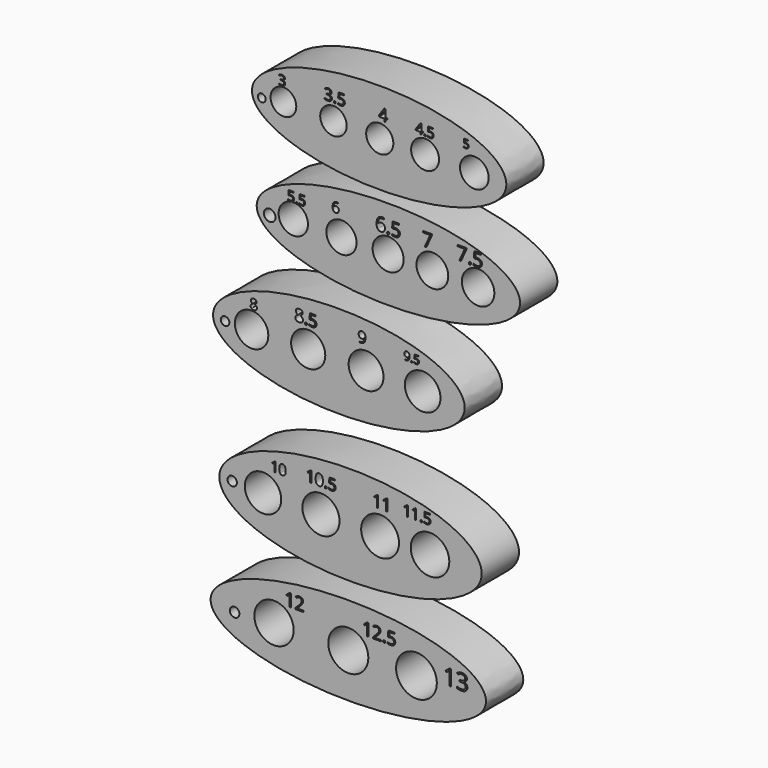
from build123d import *

# Parameters (mm, degrees)
F0_R     = 2.136468935
F0_R_2   = 7
F0_R_3   = 7.2
F0_R_4   = 7.4
F0_R_5   = 7.6
F0_R_6   = 7.8
F1_DEPTH = 25.4
F0_R_7   = 3.1544407866
F0_R_8   = 8.225
F0_R_9   = 8.45
F0_R_10  = 8.65
F0_R_11  = 8.85
F0_R_12  = 2.3340121445
F0_R_13  = 9.1
F0_R_14  = 9.3
F0_R_15  = 9.5
F0_R_16  = 9.7
F0_R_17  = 2.5272230329
F0_R_18  = 9.9
F0_R_19  = 10.1
F0_R_20  = 10.3
F0_R_21  = 10.5
F0_R_22  = 2.5984793901
F0_R_23  = 10.7
F0_R_24  = 10.9
F0_R_25  = 11.1


with BuildPart() as f1:
    # F0 (on Front) → F1 (new body)
    with BuildSketch(Plane.XZ):
        with BuildLine():
            add(Edge.make_bspline(
                [(-74.2498771352, 49.6011301875), (-74.2498771352, 6.400015037), (29.5926956492, 28.0005726122), (133.4352684336, 49.6011301875), (29.5926956492, 71.2016877628), (-74.2498771352, 92.8022453381), (-74.2498771352, 49.6011301875)],
                knots=[0, 0, 0, 2.0943951024, 2.0943951024, 4.1887902048, 4.1887902048, 6.2831853072, 6.2831853072, 6.2831853072], degree=2, weights=[1, 0.5, 1, 0.5, 1, 0.5, 1]))
        make_face()
        with Locations((-68.9354538918, 47.8157065809)):
            Circle(F0_R, mode=Mode.SUBTRACT)
        with Locations((-57.1373325878, 49.7364840567)):
            Circle(F0_R_2, mode=Mode.SUBTRACT)
        with BuildLine():
            add(Edge.make_bspline(
                [(-56.7446886804, 62.1784247059), (-56.3190353957, 61.827174231), (-56.3190353957, 61.2146487725)],
                knots=[0, 0, 0, 1, 1, 1], degree=2))
            add(Edge.make_bspline(
                [(-56.3190353957, 61.2146487725), (-56.3190353957, 60.7094017841), (-56.6022274862, 60.3887199056)],
                knots=[0, 0, 0, 1, 1, 1], degree=2))
            add(Edge.make_bspline(
                [(-56.6022274862, 60.3887199056), (-56.8854195768, 60.0680380271), (-57.4045089484, 59.959606025)],
                knots=[0, 0, 0, 1, 1, 1], degree=2))
            Line((-57.4045089484, 59.959606025), (-57.4045089484, 59.9307677266))
            add(Edge.make_bspline(
                [(-57.4045089484, 59.9307677266), (-56.770066383, 59.8523275548), (-56.4638036538, 59.5276083146)],
                knots=[0, 0, 0, 1, 1, 1], degree=2))
            add(Edge.make_bspline(
                [(-56.4638036538, 59.5276083146), (-56.1575409245, 59.2028890743), (-56.1575409245, 58.676878511)],
                knots=[0, 0, 0, 1, 1, 1], degree=2))
            add(Edge.make_bspline(
                [(-56.1575409245, 58.676878511), (-56.1575409245, 57.9236221561), (-56.680090892, 57.5175789143)],
                knots=[0, 0, 0, 1, 1, 1], degree=2))
            add(Edge.make_bspline(
                [(-56.680090892, 57.5175789143), (-57.2026408594, 57.1115356724), (-58.1646864949, 57.1115356724)],
                knots=[0, 0, 0, 1, 1, 1], degree=2))
            add(Edge.make_bspline(
                [(-58.1646864949, 57.1115356724), (-58.5834185881, 57.1115356724), (-58.9312084671, 57.174979929)],
                knots=[0, 0, 0, 1, 1, 1], degree=2))
            add(Edge.make_bspline(
                [(-58.9312084671, 57.174979929), (-59.2789983461, 57.2384241855), (-59.6066014162, 57.3964580609)],
                knots=[0, 0, 0, 1, 1, 1], degree=2))
            Line((-59.6066014162, 57.3964580609), (-59.6066014162, 57.9663028378))
            add(Edge.make_bspline(
                [(-59.6066014162, 57.9663028378), (-59.2640024309, 57.796733643), (-58.8764157001, 57.7084884499)],
                knots=[0, 0, 0, 1, 1, 1], degree=2))
            add(Edge.make_bspline(
                [(-58.8764157001, 57.7084884499), (-58.4888289692, 57.6202432567), (-58.1427693881, 57.6202432567)],
                knots=[0, 0, 0, 1, 1, 1], degree=2))
            add(Edge.make_bspline(
                [(-58.1427693881, 57.6202432567), (-56.7769875747, 57.6202432567), (-56.7769875747, 58.6907208942)],
                knots=[0, 0, 0, 1, 1, 1], degree=2))
            add(Edge.make_bspline(
                [(-56.7769875747, 58.6907208942), (-56.7769875747, 59.6504594659), (-58.2835002844, 59.6504594659)],
                knots=[0, 0, 0, 1, 1, 1], degree=2))
            Line((-58.2835002844, 59.6504594659), (-58.8025896561, 59.6504594659))
            Line((-58.8025896561, 59.6504594659), (-58.8025896561, 60.1649347098))
            Line((-58.8025896561, 60.1649347098), (-58.2765790928, 60.1649347098))
            add(Edge.make_bspline(
                [(-58.2765790928, 60.1649347098), (-57.6605930384, 60.1649347098), (-57.3001143081, 60.4371682469)],
                knots=[0, 0, 0, 1, 1, 1], degree=2))
            add(Edge.make_bspline(
                [(-57.3001143081, 60.4371682469), (-56.9396355778, 60.7094017841), (-56.9396355778, 61.1927316657)],
                knots=[0, 0, 0, 1, 1, 1], degree=2))
            add(Edge.make_bspline(
                [(-56.9396355778, 61.1927316657), (-56.9396355778, 61.5780113326), (-57.2043711573, 61.7983359326)],
                knots=[0, 0, 0, 1, 1, 1], degree=2))
            add(Edge.make_bspline(
                [(-57.2043711573, 61.7983359326), (-57.4691067369, 62.0186605326), (-57.9235983201, 62.0186605326)],
                knots=[0, 0, 0, 1, 1, 1], degree=2))
            add(Edge.make_bspline(
                [(-57.9235983201, 62.0186605326), (-58.2696579012, 62.0186605326), (-58.5759206305, 61.9246476797)],
                knots=[0, 0, 0, 1, 1, 1], degree=2))
            add(Edge.make_bspline(
                [(-58.5759206305, 61.9246476797), (-58.8821833598, 61.8306348268), (-59.2755377503, 61.5780113326)],
                knots=[0, 0, 0, 1, 1, 1], degree=2))
            Line((-59.2755377503, 61.5780113326), (-59.5777631178, 61.9817475106))
            add(Edge.make_bspline(
                [(-59.5777631178, 61.9817475106), (-59.2536206435, 62.2378316006), (-58.8302744226, 62.3837533907)],
                knots=[0, 0, 0, 1, 1, 1], degree=2))
            add(Edge.make_bspline(
                [(-58.8302744226, 62.3837533907), (-58.4069282017, 62.5296751807), (-57.9374407033, 62.5296751807)],
                knots=[0, 0, 0, 1, 1, 1], degree=2))
            add(Edge.make_bspline(
                [(-57.9374407033, 62.5296751807), (-57.1703419652, 62.5296751807), (-56.7446886804, 62.1784247059)],
                knots=[0, 0, 0, 1, 1, 1], degree=2))
        make_face(mode=Mode.SUBTRACT)
        with Locations((-29.9146188715, 49.4871671767)):
            Circle(F0_R_3, mode=Mode.SUBTRACT)
        with BuildLine():
            add(Edge.make_bspline(
                [(-29.5036788723, 58.160487771), (-29.6406609511, 58.2896048501), (-29.6406609511, 58.5845423403)],
                knots=[0, 0, 0, 1, 1, 1], degree=2))
            add(Edge.make_bspline(
                [(-29.6406609511, 58.5845423403), (-29.6406609511, 58.8598173312), (-29.5154763719, 59.0007319099)],
                knots=[0, 0, 0, 1, 1, 1], degree=2))
            add(Edge.make_bspline(
                [(-29.5154763719, 59.0007319099), (-29.3902917927, 59.1416464886), (-29.1569634671, 59.1416464886)],
                knots=[0, 0, 0, 1, 1, 1], degree=2))
            add(Edge.make_bspline(
                [(-29.1569634671, 59.1416464886), (-28.9197026416, 59.1416464886), (-28.7866530626, 59.0007319099)],
                knots=[0, 0, 0, 1, 1, 1], degree=2))
            add(Edge.make_bspline(
                [(-28.7866530626, 59.0007319099), (-28.6536034837, 58.8598173312), (-28.6536034837, 58.5845423403)],
                knots=[0, 0, 0, 1, 1, 1], degree=2))
            add(Edge.make_bspline(
                [(-28.6536034837, 58.5845423403), (-28.6536034837, 58.3184431824), (-28.7886193126, 58.1749069372)],
                knots=[0, 0, 0, 1, 1, 1], degree=2))
            add(Edge.make_bspline(
                [(-28.7886193126, 58.1749069372), (-28.9236351414, 58.0313706919), (-29.1569634671, 58.0313706919)],
                knots=[0, 0, 0, 1, 1, 1], degree=2))
            add(Edge.make_bspline(
                [(-29.1569634671, 58.0313706919), (-29.3666967935, 58.0313706919), (-29.5036788723, 58.160487771)],
                knots=[0, 0, 0, 1, 1, 1], degree=2))
        make_face(mode=Mode.SUBTRACT)
        with BuildLine():
            add(Edge.make_bspline(
                [(-31.4220833922, 63.8259092504), (-30.9383859082, 63.4267605136), (-30.9383859082, 62.7307080366)],
                knots=[0, 0, 0, 1, 1, 1], degree=2))
            add(Edge.make_bspline(
                [(-30.9383859082, 62.7307080366), (-30.9383859082, 62.1565630556), (-31.2601954809, 61.792151401)],
                knots=[0, 0, 0, 1, 1, 1], degree=2))
            add(Edge.make_bspline(
                [(-31.2601954809, 61.792151401), (-31.5820050536, 61.4277397464), (-32.1718800341, 61.3045214171)],
                knots=[0, 0, 0, 1, 1, 1], degree=2))
            Line((-32.1718800341, 61.3045214171), (-32.1718800341, 61.2717505848))
            add(Edge.make_bspline(
                [(-32.1718800341, 61.2717505848), (-31.4509217246, 61.1826139211), (-31.1028954861, 60.81361435)],
                knots=[0, 0, 0, 1, 1, 1], degree=2))
            add(Edge.make_bspline(
                [(-31.1028954861, 60.81361435), (-30.7548692476, 60.4446147788), (-30.7548692476, 59.8468747986)],
                knots=[0, 0, 0, 1, 1, 1], degree=2))
            add(Edge.make_bspline(
                [(-30.7548692476, 59.8468747986), (-30.7548692476, 58.9909006602), (-31.348676728, 58.5294873421)],
                knots=[0, 0, 0, 1, 1, 1], degree=2))
            add(Edge.make_bspline(
                [(-31.348676728, 58.5294873421), (-31.9424842083, 58.068074024), (-33.0357191722, 58.068074024)],
                knots=[0, 0, 0, 1, 1, 1], degree=2))
            add(Edge.make_bspline(
                [(-33.0357191722, 58.068074024), (-33.5115516565, 58.068074024), (-33.9067678934, 58.140169855)],
                knots=[0, 0, 0, 1, 1, 1], degree=2))
            add(Edge.make_bspline(
                [(-33.9067678934, 58.140169855), (-34.3019841304, 58.212265686), (-34.6742607847, 58.3918498467)],
                knots=[0, 0, 0, 1, 1, 1], degree=2))
            Line((-34.6742607847, 58.3918498467), (-34.6742607847, 59.0394014919))
            add(Edge.make_bspline(
                [(-34.6742607847, 59.0394014919), (-34.2849432976, 58.8467089983), (-33.8445033121, 58.7464302516)],
                knots=[0, 0, 0, 1, 1, 1], degree=2))
            add(Edge.make_bspline(
                [(-33.8445033121, 58.7464302516), (-33.4040633267, 58.6461515049), (-33.0108133397, 58.6461515049)],
                knots=[0, 0, 0, 1, 1, 1], degree=2))
            add(Edge.make_bspline(
                [(-33.0108133397, 58.6461515049), (-31.4587867243, 58.6461515049), (-31.4587867243, 59.8626047981)],
                knots=[0, 0, 0, 1, 1, 1], degree=2))
            add(Edge.make_bspline(
                [(-31.4587867243, 59.8626047981), (-31.4587867243, 60.9532180954), (-33.1707350011, 60.9532180954)],
                knots=[0, 0, 0, 1, 1, 1], degree=2))
            Line((-33.1707350011, 60.9532180954), (-33.7606099816, 60.9532180954))
            Line((-33.7606099816, 60.9532180954), (-33.7606099816, 61.5378497427))
            Line((-33.7606099816, 61.5378497427), (-33.1628700013, 61.5378497427))
            add(Edge.make_bspline(
                [(-33.1628700013, 61.5378497427), (-32.4628850245, 61.5378497427), (-32.0532496213, 61.8472063992)],
                knots=[0, 0, 0, 1, 1, 1], degree=2))
            add(Edge.make_bspline(
                [(-32.0532496213, 61.8472063992), (-31.6436142182, 62.1565630556), (-31.6436142182, 62.7058022041)],
                knots=[0, 0, 0, 1, 1, 1], degree=2))
            add(Edge.make_bspline(
                [(-31.6436142182, 62.7058022041), (-31.6436142182, 63.143620523), (-31.9444504583, 63.3939896814)],
                knots=[0, 0, 0, 1, 1, 1], degree=2))
            add(Edge.make_bspline(
                [(-31.9444504583, 63.3939896814), (-32.2452866983, 63.6443588398), (-32.7617550146, 63.6443588398)],
                knots=[0, 0, 0, 1, 1, 1], degree=2))
            add(Edge.make_bspline(
                [(-32.7617550146, 63.6443588398), (-33.1550050016, 63.6443588398), (-33.5030312401, 63.5375259266)],
                knots=[0, 0, 0, 1, 1, 1], degree=2))
            add(Edge.make_bspline(
                [(-33.5030312401, 63.5375259266), (-33.8510574786, 63.4306930135), (-34.2980516305, 63.143620523)],
                knots=[0, 0, 0, 1, 1, 1], degree=2))
            Line((-34.2980516305, 63.143620523), (-34.6414899525, 63.6024121745))
            add(Edge.make_bspline(
                [(-34.6414899525, 63.6024121745), (-34.273145798, 63.8934171649), (-33.7920699805, 64.0592375761)],
                knots=[0, 0, 0, 1, 1, 1], degree=2))
            add(Edge.make_bspline(
                [(-33.7920699805, 64.0592375761), (-33.3109941631, 64.2250579872), (-32.7774850141, 64.2250579872)],
                knots=[0, 0, 0, 1, 1, 1], degree=2))
            add(Edge.make_bspline(
                [(-32.7774850141, 64.2250579872), (-31.9057808762, 64.2250579872), (-31.4220833922, 63.8259092504)],
                knots=[0, 0, 0, 1, 1, 1], degree=2))
        make_face(mode=Mode.SUBTRACT)
        with BuildLine():
            add(Edge.make_bspline(
                [(-26.6873535487, 61.7148122369), (-26.2167643976, 61.8091922337), (-25.748796913, 61.8091922337)],
                knots=[0, 0, 0, 1, 1, 1], degree=2))
            add(Edge.make_bspline(
                [(-25.748796913, 61.8091922337), (-24.8023752776, 61.8091922337), (-24.2596902956, 61.3399139159)],
                knots=[0, 0, 0, 1, 1, 1], degree=2))
            add(Edge.make_bspline(
                [(-24.2596902956, 61.3399139159), (-23.7170053135, 60.8706355981), (-23.7170053135, 60.0552972917)],
                knots=[0, 0, 0, 1, 1, 1], degree=2))
            add(Edge.make_bspline(
                [(-23.7170053135, 60.0552972917), (-23.7170053135, 59.1259164891), (-24.3088465439, 58.5969952566)],
                knots=[0, 0, 0, 1, 1, 1], degree=2))
            add(Edge.make_bspline(
                [(-24.3088465439, 58.5969952566), (-24.9006877744, 58.068074024), (-25.9414894067, 58.068074024)],
                knots=[0, 0, 0, 1, 1, 1], degree=2))
            add(Edge.make_bspline(
                [(-25.9414894067, 58.068074024), (-26.9534527065, 58.068074024), (-27.4856510223, 58.3918498467)],
                knots=[0, 0, 0, 1, 1, 1], degree=2))
            Line((-27.4856510223, 58.3918498467), (-27.4856510223, 59.0472664917))
            add(Edge.make_bspline(
                [(-27.4856510223, 59.0472664917), (-27.1998893651, 58.8637498311), (-26.7738685458, 58.7588831679)],
                knots=[0, 0, 0, 1, 1, 1], degree=2))
            add(Edge.make_bspline(
                [(-26.7738685458, 58.7588831679), (-26.3478477266, 58.6540165047), (-25.9336244069, 58.6540165047)],
                knots=[0, 0, 0, 1, 1, 1], degree=2))
            add(Edge.make_bspline(
                [(-25.9336244069, 58.6540165047), (-25.2126660974, 58.6540165047), (-24.8135173606, 58.9941777434)],
                knots=[0, 0, 0, 1, 1, 1], degree=2))
            add(Edge.make_bspline(
                [(-24.8135173606, 58.9941777434), (-24.4143686238, 59.3343389822), (-24.4143686238, 59.9779581276)],
                knots=[0, 0, 0, 1, 1, 1], degree=2))
            add(Edge.make_bspline(
                [(-24.4143686238, 59.9779581276), (-24.4143686238, 61.2311147528), (-25.9493544064, 61.2311147528)],
                knots=[0, 0, 0, 1, 1, 1], degree=2))
            add(Edge.make_bspline(
                [(-25.9493544064, 61.2311147528), (-26.3386718935, 61.2311147528), (-26.9901560387, 61.1118289235)],
                knots=[0, 0, 0, 1, 1, 1], degree=2))
            Line((-26.9901560387, 61.1118289235), (-27.3427701937, 61.3372922493))
            Line((-27.3427701937, 61.3372922493), (-27.1173068678, 64.1398538234))
            Line((-27.1173068678, 64.1398538234), (-24.1390936329, 64.1398538234))
            Line((-24.1390936329, 64.1398538234), (-24.1390936329, 63.5132755108))
            Line((-24.1390936329, 63.5132755108), (-26.535296887, 63.5132755108))
            Line((-26.535296887, 63.5132755108), (-26.6873535487, 61.7148122369))
        make_face(mode=Mode.SUBTRACT)
        with Locations((-4.6957170294, 49.2425088413)):
            Circle(F0_R_4, mode=Mode.SUBTRACT)
        Polygon((-0.5657551648, 60.2255465476), (-0.5657551648, 59.5820852517), (-1.490049145, 59.5820852517), (-1.490049145, 58.1506565213), (-2.1675920774, 58.1506565213), (-2.1675920774, 59.5820852517), (-5.1967679238, 59.5820852517), (-5.1967679238, 60.1996445039), (-2.2398451466, 64.4134980329), (-1.490049145, 64.4134980329), (-1.490049145, 60.2255465476), align=None, mode=Mode.SUBTRACT)
        with Locations((19.9792224744, 49.6208461123)):
            Circle(F0_R_5, mode=Mode.SUBTRACT)
        Polygon((18.7856617025, 60.1479470077), (18.7856617025, 59.6034799334), (18.0035670492, 59.6034799334), (18.0035670492, 58.3922713995), (17.4302616765, 58.3922713995), (17.4302616765, 59.6034799334), (14.8671137124, 59.6034799334), (14.8671137124, 60.1260299009), (17.3691244838, 63.6915971182), (18.0035670492, 63.6915971182), (18.0035670492, 60.1479470077), align=None, mode=Mode.SUBTRACT)
        with BuildLine():
            add(Edge.make_bspline(
                [(19.6017855479, 58.400922889), (19.4812414605, 58.5145457848), (19.4812414605, 58.7740904707)],
                knots=[0, 0, 0, 1, 1, 1], degree=2))
            add(Edge.make_bspline(
                [(19.4812414605, 58.7740904707), (19.4812414605, 59.0163321774), (19.5914037605, 59.1403368607)],
                knots=[0, 0, 0, 1, 1, 1], degree=2))
            add(Edge.make_bspline(
                [(19.5914037605, 59.1403368607), (19.7015660605, 59.2643415439), (19.9068947453, 59.2643415439)],
                knots=[0, 0, 0, 1, 1, 1], degree=2))
            add(Edge.make_bspline(
                [(19.9068947453, 59.2643415439), (20.1156840259, 59.2643415439), (20.2327675175, 59.1403368607)],
                knots=[0, 0, 0, 1, 1, 1], degree=2))
            add(Edge.make_bspline(
                [(20.2327675175, 59.1403368607), (20.3498510091, 59.0163321774), (20.3498510091, 58.7740904707)],
                knots=[0, 0, 0, 1, 1, 1], degree=2))
            add(Edge.make_bspline(
                [(20.3498510091, 58.7740904707), (20.3498510091, 58.5399234874), (20.2310372196, 58.4136117403)],
                knots=[0, 0, 0, 1, 1, 1], degree=2))
            add(Edge.make_bspline(
                [(20.2310372196, 58.4136117403), (20.1122234301, 58.2872999932), (19.9068947453, 58.2872999932)],
                knots=[0, 0, 0, 1, 1, 1], degree=2))
            add(Edge.make_bspline(
                [(19.9068947453, 58.2872999932), (19.7223296353, 58.2872999932), (19.6017855479, 58.400922889)],
                knots=[0, 0, 0, 1, 1, 1], degree=2))
        make_face(mode=Mode.SUBTRACT)
        with BuildLine():
            add(Edge.make_bspline(
                [(22.0801489146, 61.5287247363), (22.49426688, 61.6117790358), (22.9060777815, 61.6117790358)],
                knots=[0, 0, 0, 1, 1, 1], degree=2))
            add(Edge.make_bspline(
                [(22.9060777815, 61.6117790358), (23.7389278401, 61.6117790358), (24.216490062, 61.1988146023)],
                knots=[0, 0, 0, 1, 1, 1], degree=2))
            add(Edge.make_bspline(
                [(24.216490062, 61.1988146023), (24.6940522839, 60.7858501688), (24.6940522839, 60.068353304)],
                knots=[0, 0, 0, 1, 1, 1], degree=2))
            add(Edge.make_bspline(
                [(24.6940522839, 60.068353304), (24.6940522839, 59.2504991606), (24.1732326144, 58.7850490241)],
                knots=[0, 0, 0, 1, 1, 1], degree=2))
            add(Edge.make_bspline(
                [(24.1732326144, 58.7850490241), (23.6524129448, 58.3195988875), (22.7365085868, 58.3195988875)],
                knots=[0, 0, 0, 1, 1, 1], degree=2))
            add(Edge.make_bspline(
                [(22.7365085868, 58.3195988875), (21.8459819314, 58.3195988875), (21.377647965, 58.6045212759)],
                knots=[0, 0, 0, 1, 1, 1], degree=2))
            Line((21.377647965, 58.6045212759), (21.377647965, 59.1812872444))
            add(Edge.make_bspline(
                [(21.377647965, 59.1812872444), (21.6291179273, 59.0197927732), (22.0040158068, 58.9275102183)],
                knots=[0, 0, 0, 1, 1, 1], degree=2))
            add(Edge.make_bspline(
                [(22.0040158068, 58.9275102183), (22.3789136863, 58.8352276633), (22.7434297784, 58.8352276633)],
                knots=[0, 0, 0, 1, 1, 1], degree=2))
            add(Edge.make_bspline(
                [(22.7434297784, 58.8352276633), (23.3778723438, 58.8352276633), (23.7291228186, 59.134569201)],
                knots=[0, 0, 0, 1, 1, 1], degree=2))
            add(Edge.make_bspline(
                [(23.7291228186, 59.134569201), (24.0803732934, 59.4339107386), (24.0803732934, 60.0002949197)],
                knots=[0, 0, 0, 1, 1, 1], degree=2))
            add(Edge.make_bspline(
                [(24.0803732934, 60.0002949197), (24.0803732934, 61.1030714515), (22.7295873952, 61.1030714515)],
                knots=[0, 0, 0, 1, 1, 1], degree=2))
            add(Edge.make_bspline(
                [(22.7295873952, 61.1030714515), (22.3869884099, 61.1030714515), (21.8136830372, 60.9981000453)],
                knots=[0, 0, 0, 1, 1, 1], degree=2))
            Line((21.8136830372, 60.9981000453), (21.5033829461, 61.1965075384))
            Line((21.5033829461, 61.1965075384), (21.7017904393, 63.6627588198))
            Line((21.7017904393, 63.6627588198), (24.3226150002, 63.6627588198))
            Line((24.3226150002, 63.6627588198), (24.3226150002, 63.1113705539))
            Line((24.3226150002, 63.1113705539), (22.2139586193, 63.1113705539))
            Line((22.2139586193, 63.1113705539), (22.0801489146, 61.5287247363))
        make_face(mode=Mode.SUBTRACT)
        with Locations((46.8104465027, 49.6208461123)):
            Circle(F0_R_6, mode=Mode.SUBTRACT)
        with BuildLine():
            add(Edge.make_bspline(
                [(41.5835945322, 62.3727190387), (41.9291500455, 62.4420226514), (42.2727804584, 62.4420226514)],
                knots=[0, 0, 0, 1, 1, 1], degree=2))
            add(Edge.make_bspline(
                [(42.2727804584, 62.4420226514), (42.9677416857, 62.4420226514), (43.3662374586, 62.0974296883)],
                knots=[0, 0, 0, 1, 1, 1], degree=2))
            add(Edge.make_bspline(
                [(43.3662374586, 62.0974296883), (43.7647332316, 61.7528367252), (43.7647332316, 61.1541305156)],
                knots=[0, 0, 0, 1, 1, 1], degree=2))
            add(Edge.make_bspline(
                [(43.7647332316, 61.1541305156), (43.7647332316, 60.4716824406), (43.330141827, 60.0832934445)],
                knots=[0, 0, 0, 1, 1, 1], degree=2))
            add(Edge.make_bspline(
                [(43.330141827, 60.0832934445), (42.8955504224, 59.6949044484), (42.1312855825, 59.6949044484)],
                knots=[0, 0, 0, 1, 1, 1], degree=2))
            add(Edge.make_bspline(
                [(42.1312855825, 59.6949044484), (41.3881968464, 59.6949044484), (40.9974014749, 59.9326543419)],
                knots=[0, 0, 0, 1, 1, 1], degree=2))
            Line((40.9974014749, 59.9326543419), (40.9974014749, 60.4139294301))
            add(Edge.make_bspline(
                [(40.9974014749, 60.4139294301), (41.2072374133, 60.2791724054), (41.5200662206, 60.2021683913)],
                knots=[0, 0, 0, 1, 1, 1], degree=2))
            add(Edge.make_bspline(
                [(41.5200662206, 60.2021683913), (41.8328950279, 60.1251643772), (42.1370608836, 60.1251643772)],
                knots=[0, 0, 0, 1, 1, 1], degree=2))
            add(Edge.make_bspline(
                [(42.1370608836, 60.1251643772), (42.6664634805, 60.1251643772), (42.9595600092, 60.3749461479)],
                knots=[0, 0, 0, 1, 1, 1], degree=2))
            add(Edge.make_bspline(
                [(42.9595600092, 60.3749461479), (43.2526565378, 60.6247279187), (43.2526565378, 61.0973400552)],
                knots=[0, 0, 0, 1, 1, 1], degree=2))
            add(Edge.make_bspline(
                [(43.2526565378, 61.0973400552), (43.2526565378, 62.0175380237), (42.1255102814, 62.0175380237)],
                knots=[0, 0, 0, 1, 1, 1], degree=2))
            add(Edge.make_bspline(
                [(42.1255102814, 62.0175380237), (41.8396328791, 62.0175380237), (41.3612454415, 61.9299459577)],
                knots=[0, 0, 0, 1, 1, 1], degree=2))
            Line((41.3612454415, 61.9299459577), (41.1023194441, 62.095504588))
            Line((41.1023194441, 62.095504588), (41.2678780744, 64.1534368648))
            Line((41.2678780744, 64.1534368648), (43.4547920749, 64.1534368648))
            Line((43.4547920749, 64.1534368648), (43.4547920749, 63.6933378806))
            Line((43.4547920749, 63.6933378806), (41.6952503527, 63.6933378806))
            Line((41.6952503527, 63.6933378806), (41.5835945322, 62.3727190387))
        make_face(mode=Mode.SUBTRACT)
    extrude(amount=F1_DEPTH)


with BuildPart() as f1b:
    # F0 (on Front) → F1, piece 2 (new body)
    with BuildSketch(Plane.XZ):
        with BuildLine():
            add(Edge.make_bspline(
                [(-71.6832986265, -4.7536236234), (-71.6832986265, -47.1143562515), (35.8416493133, -25.9339899375), (143.3665972531, -4.7536236234), (35.8416493133, 16.4267426907), (-71.6832986265, 37.6071090047), (-71.6832986265, -4.7536236234)],
                knots=[0, 0, 0, 2.0943951024, 2.0943951024, 4.1887902048, 4.1887902048, 6.2831853072, 6.2831853072, 6.2831853072], degree=2, weights=[1, 0.5, 1, 0.5, 1, 0.5, 1]))
        make_face()
        with Locations((-64.5886436105, -7.0209745318)):
            Circle(F0_R_7, mode=Mode.SUBTRACT)
        with BuildLine():
            ThreePointArc((-52.4649288701, 3.3297638507), (-46.3536171258, 1.2647660314), (-43.7528454239, -4.6384817006))
            ThreePointArc((-43.7528454239, -4.6384817006), (-56.8302853383, -10.8206822729), (-53.3077464029, 3.2089562855))
            add(Edge.make_bspline(
                [(-53.3077464029, 3.2089562855), (-54.1693614709, 3.2120694111), (-54.6249166315, 3.4892175014)],
                knots=[0.0112327152, 0.0112327152, 0.0112327152, 1, 1, 1], degree=2))
            Line((-54.6249166315, 3.4892175014), (-54.6249166315, 4.0566194893))
            add(Edge.make_bspline(
                [(-54.6249166315, 4.0566194893), (-54.3775293648, 3.8977469327), (-54.0087180727, 3.8069626147)],
                knots=[0, 0, 0, 1, 1, 1], degree=2))
            add(Edge.make_bspline(
                [(-54.0087180727, 3.8069626147), (-53.6399067805, 3.7161782966), (-53.2813087242, 3.7161782966)],
                knots=[0, 0, 0, 1, 1, 1], degree=2))
            add(Edge.make_bspline(
                [(-53.2813087242, 3.7161782966), (-52.6571665375, 3.7161782966), (-52.3116187268, 4.0106599283)],
                knots=[0, 0, 0, 1, 1, 1], degree=2))
            add(Edge.make_bspline(
                [(-52.3116187268, 4.0106599283), (-51.9660709162, 4.3051415601), (-51.9660709162, 4.8623303122)],
                knots=[0, 0, 0, 1, 1, 1], degree=2))
            add(Edge.make_bspline(
                [(-51.9660709162, 4.8623303122), (-51.9660709162, 5.9472029131), (-53.2949263719, 5.9472029131)],
                knots=[0, 0, 0, 1, 1, 1], degree=2))
            add(Edge.make_bspline(
                [(-53.2949263719, 5.9472029131), (-53.6319631527, 5.9472029131), (-54.1959607287, 5.8439357513)],
                knots=[0, 0, 0, 1, 1, 1], degree=2))
            Line((-54.1959607287, 5.8439357513), (-54.5012229982, 6.0391220351))
            Line((-54.5012229982, 6.0391220351), (-54.3060367143, 8.4653329354))
            Line((-54.3060367143, 8.4653329354), (-51.7277620813, 8.4653329354))
            Line((-51.7277620813, 8.4653329354), (-51.7277620813, 7.922896635))
            Line((-51.7277620813, 7.922896635), (-53.8021837491, 7.922896635))
            Line((-53.8021837491, 7.922896635), (-53.9338210103, 6.3659455802))
            add(Edge.make_bspline(
                [(-53.9338210103, 6.3659455802), (-53.5264263829, 6.4476514664), (-53.1213013636, 6.4476514664)],
                knots=[0, 0, 0, 1, 1, 1], degree=2))
            add(Edge.make_bspline(
                [(-53.1213013636, 6.4476514664), (-52.301972893, 6.4476514664), (-51.832164047, 6.0413916431)],
                knots=[0, 0, 0, 1, 1, 1], degree=2))
            add(Edge.make_bspline(
                [(-51.832164047, 6.0413916431), (-51.362355201, 5.6351318197), (-51.362355201, 4.9292837468)],
                knots=[0, 0, 0, 1, 1, 1], degree=2))
            add(Edge.make_bspline(
                [(-51.362355201, 4.9292837468), (-51.362355201, 4.1247077279), (-51.8747191961, 3.6668143237)],
                knots=[0, 0, 0, 1, 1, 1], degree=2))
            add(Edge.make_bspline(
                [(-51.8747191961, 3.6668143237), (-52.123870373, 3.4441509796), (-52.4649288701, 3.3297638507)],
                knots=[0, 0, 0, 0.4862776839, 0.4862776839, 0.4862776839], degree=2))
        make_face(mode=Mode.SUBTRACT)
        with Locations((-25.5409889905, -4.8742699142)):
            Circle(F0_R_8, mode=Mode.SUBTRACT)
        with BuildLine():
            add(Edge.make_bspline(
                [(-50.2871284339, 3.2889245997), (-50.4057154494, 3.4007027913), (-50.4057154494, 3.6560336859)],
                knots=[0, 0, 0, 1, 1, 1], degree=2))
            add(Edge.make_bspline(
                [(-50.4057154494, 3.6560336859), (-50.4057154494, 3.8943425208), (-50.2973416697, 4.0163339482)],
                knots=[0, 0, 0, 1, 1, 1], degree=2))
            add(Edge.make_bspline(
                [(-50.2973416697, 4.0163339482), (-50.18896789, 4.1383253756), (-49.9869727823, 4.1383253756)],
                knots=[0, 0, 0, 1, 1, 1], degree=2))
            add(Edge.make_bspline(
                [(-49.9869727823, 4.1383253756), (-49.7815732627, 4.1383253756), (-49.6663906592, 4.0163339482)],
                knots=[0, 0, 0, 1, 1, 1], degree=2))
            add(Edge.make_bspline(
                [(-49.6663906592, 4.0163339482), (-49.5512080556, 3.8943425208), (-49.5512080556, 3.6560336859)],
                knots=[0, 0, 0, 1, 1, 1], degree=2))
            add(Edge.make_bspline(
                [(-49.5512080556, 3.6560336859), (-49.5512080556, 3.4256684788), (-49.6680928651, 3.3014074434)],
                knots=[0, 0, 0, 1, 1, 1], degree=2))
            add(Edge.make_bspline(
                [(-49.6680928651, 3.3014074434), (-49.7849776746, 3.1771464081), (-49.9869727823, 3.1771464081)],
                knots=[0, 0, 0, 1, 1, 1], degree=2))
            add(Edge.make_bspline(
                [(-49.9869727823, 3.1771464081), (-50.1685414185, 3.1771464081), (-50.2871284339, 3.2889245997)],
                knots=[0, 0, 0, 1, 1, 1], degree=2))
        make_face(mode=Mode.SUBTRACT)
        with BuildLine():
            add(Edge.make_bspline(
                [(-47.8490020919, 6.3659455802), (-47.4416074646, 6.4476514664), (-47.0364824452, 6.4476514664)],
                knots=[0, 0, 0, 1, 1, 1], degree=2))
            add(Edge.make_bspline(
                [(-47.0364824452, 6.4476514664), (-46.2171539746, 6.4476514664), (-45.7473451287, 6.0413916431)],
                knots=[0, 0, 0, 1, 1, 1], degree=2))
            add(Edge.make_bspline(
                [(-45.7473451287, 6.0413916431), (-45.2775362827, 5.6351318197), (-45.2775362827, 4.9292837468)],
                knots=[0, 0, 0, 1, 1, 1], degree=2))
            add(Edge.make_bspline(
                [(-45.2775362827, 4.9292837468), (-45.2775362827, 4.1247077279), (-45.7899002777, 3.6668143237)],
                knots=[0, 0, 0, 1, 1, 1], degree=2))
            add(Edge.make_bspline(
                [(-45.7899002777, 3.6668143237), (-46.3022642728, 3.2089209194), (-47.2032986296, 3.2089209194)],
                knots=[0, 0, 0, 1, 1, 1], degree=2))
            add(Edge.make_bspline(
                [(-47.2032986296, 3.2089209194), (-48.079367299, 3.2089209194), (-48.5400977132, 3.4892175014)],
                knots=[0, 0, 0, 1, 1, 1], degree=2))
            Line((-48.5400977132, 3.4892175014), (-48.5400977132, 4.0566194893))
            add(Edge.make_bspline(
                [(-48.5400977132, 4.0566194893), (-48.2927104464, 3.8977469327), (-47.9238991543, 3.8069626147)],
                knots=[0, 0, 0, 1, 1, 1], degree=2))
            add(Edge.make_bspline(
                [(-47.9238991543, 3.8069626147), (-47.5550878621, 3.7161782966), (-47.1964898058, 3.7161782966)],
                knots=[0, 0, 0, 1, 1, 1], degree=2))
            add(Edge.make_bspline(
                [(-47.1964898058, 3.7161782966), (-46.5723476191, 3.7161782966), (-46.2267998084, 4.0106599283)],
                knots=[0, 0, 0, 1, 1, 1], degree=2))
            add(Edge.make_bspline(
                [(-46.2267998084, 4.0106599283), (-45.8812519978, 4.3051415601), (-45.8812519978, 4.8623303122)],
                knots=[0, 0, 0, 1, 1, 1], degree=2))
            add(Edge.make_bspline(
                [(-45.8812519978, 4.8623303122), (-45.8812519978, 5.9472029131), (-47.2101074535, 5.9472029131)],
                knots=[0, 0, 0, 1, 1, 1], degree=2))
            add(Edge.make_bspline(
                [(-47.2101074535, 5.9472029131), (-47.5471442343, 5.9472029131), (-48.1111418103, 5.8439357513)],
                knots=[0, 0, 0, 1, 1, 1], degree=2))
            Line((-48.1111418103, 5.8439357513), (-48.4164040798, 6.0391220351))
            Line((-48.4164040798, 6.0391220351), (-48.221217796, 8.4653329354))
            Line((-48.221217796, 8.4653329354), (-45.6429431629, 8.4653329354))
            Line((-45.6429431629, 8.4653329354), (-45.6429431629, 7.922896635))
            Line((-45.6429431629, 7.922896635), (-47.7173648307, 7.922896635))
            Line((-47.7173648307, 7.922896635), (-47.8490020919, 6.3659455802))
        make_face(mode=Mode.SUBTRACT)
        with BuildLine():
            add(Edge.make_bspline(
                [(-29.8944641145, 6.4283589648), (-30.3659753554, 7.0332097263), (-30.3659753554, 8.1112739354)],
                knots=[0, 0, 0, 1, 1, 1], degree=2))
            add(Edge.make_bspline(
                [(-30.3659753554, 8.1112739354), (-30.3659753554, 9.6398555033), (-29.771905236, 10.3967700585)],
                knots=[0, 0, 0, 1, 1, 1], degree=2))
            add(Edge.make_bspline(
                [(-29.771905236, 10.3967700585), (-29.1778351166, 11.1536846137), (-28.0146605752, 11.1536846137)],
                knots=[0, 0, 0, 1, 1, 1], degree=2))
            add(Edge.make_bspline(
                [(-28.0146605752, 11.1536846137), (-27.6140746112, 11.1536846137), (-27.3837093118, 11.0867311523)],
                knots=[0, 0, 0, 1, 1, 1], degree=2))
            Line((-27.3837093118, 11.0867311523), (-27.3837093118, 10.5794735719))
            add(Edge.make_bspline(
                [(-27.3837093118, 10.5794735719), (-27.6571971796, 10.6679883174), (-28.0078517486, 10.6679883174)],
                knots=[0, 0, 0, 1, 1, 1], degree=2))
            add(Edge.make_bspline(
                [(-28.0078517486, 10.6679883174), (-28.8419330051, 10.6679883174), (-29.281669722, 10.1488152904)],
                knots=[0, 0, 0, 1, 1, 1], degree=2))
            add(Edge.make_bspline(
                [(-29.281669722, 10.1488152904), (-29.7214064388, 9.6296422635), (-29.7633942027, 8.5152643126)],
                knots=[0, 0, 0, 1, 1, 1], degree=2))
            Line((-29.7633942027, 8.5152643126), (-29.7214064388, 8.5152643126))
            add(Edge.make_bspline(
                [(-29.7214064388, 8.5152643126), (-29.3310337147, 9.1257890963), (-28.4867392184, 9.1257890963)],
                knots=[0, 0, 0, 1, 1, 1], degree=2))
            add(Edge.make_bspline(
                [(-28.4867392184, 9.1257890963), (-27.7876996891, 9.1257890963), (-27.3854115185, 8.7036418481)],
                knots=[0, 0, 0, 1, 1, 1], degree=2))
            add(Edge.make_bspline(
                [(-27.3854115185, 8.7036418481), (-26.9831233478, 8.2814945999), (-26.9831233478, 7.5586241777)],
                knots=[0, 0, 0, 1, 1, 1], degree=2))
            add(Edge.make_bspline(
                [(-26.9831233478, 7.5586241777), (-26.9831233478, 6.7495086187), (-27.4245622713, 6.286508411)],
                knots=[0, 0, 0, 1, 1, 1], degree=2))
            add(Edge.make_bspline(
                [(-27.4245622713, 6.286508411), (-27.8660011948, 5.8235082033), (-28.6183765323, 5.8235082033)],
                knots=[0, 0, 0, 1, 1, 1], degree=2))
            add(Edge.make_bspline(
                [(-28.6183765323, 5.8235082033), (-29.4229528736, 5.8235082033), (-29.8944641145, 6.4283589648)],
                knots=[0, 0, 0, 1, 1, 1], degree=2))
        make_face(mode=Mode.SUBTRACT)
        with Locations((-0.1301338792, -4.6653512359)):
            Circle(F0_R_9, mode=Mode.SUBTRACT)
        with Locations((23.9531567078, -4.6653512359)):
            Circle(F0_R_10, mode=Mode.SUBTRACT)
        with Locations((48.8504094048, -4.6653512359)):
            Circle(F0_R_11, mode=Mode.SUBTRACT)
        with BuildLine():
            add(Edge.make_bspline(
                [(-5.7913023793, 5.5691998496), (-6.4278424034, 6.3857481837), (-6.4278424034, 7.8411345203)],
                knots=[0, 0, 0, 1, 1, 1], degree=2))
            add(Edge.make_bspline(
                [(-6.4278424034, 7.8411345203), (-6.4278424034, 9.904719147), (-5.6258479326, 10.9265535539)],
                knots=[0, 0, 0, 1, 1, 1], degree=2))
            add(Edge.make_bspline(
                [(-5.6258479326, 10.9265535539), (-4.8238534619, 11.9483879607), (-3.2535682039, 11.9483879607)],
                knots=[0, 0, 0, 1, 1, 1], degree=2))
            add(Edge.make_bspline(
                [(-3.2535682039, 11.9483879607), (-2.712777281, 11.9483879607), (-2.4017842006, 11.8580008093)],
                knots=[0, 0, 0, 1, 1, 1], degree=2))
            Line((-2.4017842006, 11.8580008093), (-2.4017842006, 11.1732032383))
            add(Edge.make_bspline(
                [(-2.4017842006, 11.1732032383), (-2.7709927344, 11.2926981164), (-3.2443762902, 11.2926981164)],
                knots=[0, 0, 0, 1, 1, 1], degree=2))
            add(Edge.make_bspline(
                [(-3.2443762902, 11.2926981164), (-4.3703857191, 11.2926981164), (-4.9640301459, 10.5918146965)],
                knots=[0, 0, 0, 1, 1, 1], degree=2))
            add(Edge.make_bspline(
                [(-4.9640301459, 10.5918146965), (-5.5576745726, 9.8909312765), (-5.6143580405, 8.3865214001)],
                knots=[0, 0, 0, 1, 1, 1], degree=2))
            Line((-5.6143580405, 8.3865214001), (-5.5576745726, 8.3865214001))
            add(Edge.make_bspline(
                [(-5.5576745726, 8.3865214001), (-5.0306715202, 9.2107296623), (-3.8908742208, 9.2107296623)],
                knots=[0, 0, 0, 1, 1, 1], degree=2))
            add(Edge.make_bspline(
                [(-3.8908742208, 9.2107296623), (-2.9471710805, 9.2107296623), (-2.4040821791, 8.6408310126)],
                knots=[0, 0, 0, 1, 1, 1], degree=2))
            add(Edge.make_bspline(
                [(-2.4040821791, 8.6408310126), (-1.8609932777, 8.0709323629), (-1.8609932777, 7.0950575246)],
                knots=[0, 0, 0, 1, 1, 1], degree=2))
            add(Edge.make_bspline(
                [(-1.8609932777, 7.0950575246), (-1.8609932777, 6.0027517793), (-2.4569356829, 5.3777016474)],
                knots=[0, 0, 0, 1, 1, 1], degree=2))
            add(Edge.make_bspline(
                [(-2.4569356829, 5.3777016474), (-3.0528780881, 4.7526515154), (-4.0685845524, 4.7526515154)],
                knots=[0, 0, 0, 1, 1, 1], degree=2))
            add(Edge.make_bspline(
                [(-4.0685845524, 4.7526515154), (-5.1547623552, 4.7526515154), (-5.7913023793, 5.5691998496)],
                knots=[0, 0, 0, 1, 1, 1], degree=2))
        make_face(mode=Mode.SUBTRACT)
        with BuildLine():
            add(Edge.make_bspline(
                [(-0.4952280997, 4.8606565015), (-0.6553205967, 5.0115570848), (-0.6553205967, 5.3562538487)],
                knots=[0, 0, 0, 1, 1, 1], degree=2))
            add(Edge.make_bspline(
                [(-0.6553205967, 5.3562538487), (-0.6553205967, 5.6779708284), (-0.5090159702, 5.8426592823)],
                knots=[0, 0, 0, 1, 1, 1], degree=2))
            add(Edge.make_bspline(
                [(-0.5090159702, 5.8426592823), (-0.3627113438, 6.0073477362), (-0.0900179039, 6.0073477362)],
                knots=[0, 0, 0, 1, 1, 1], degree=2))
            add(Edge.make_bspline(
                [(-0.0900179039, 6.0073477362), (0.1872714929, 6.0073477362), (0.3427680331, 5.8426592823)],
                knots=[0, 0, 0, 1, 1, 1], degree=2))
            add(Edge.make_bspline(
                [(0.3427680331, 5.8426592823), (0.4982645733, 5.6779708284), (0.4982645733, 5.3562538487)],
                knots=[0, 0, 0, 1, 1, 1], degree=2))
            add(Edge.make_bspline(
                [(0.4982645733, 5.3562538487), (0.4982645733, 5.0452607684), (0.3404700547, 4.8775083433)],
                knots=[0, 0, 0, 1, 1, 1], degree=2))
            add(Edge.make_bspline(
                [(0.3404700547, 4.8775083433), (0.1826755361, 4.7097559182), (-0.0900179039, 4.7097559182)],
                knots=[0, 0, 0, 1, 1, 1], degree=2))
            add(Edge.make_bspline(
                [(-0.0900179039, 4.7097559182), (-0.3351356027, 4.7097559182), (-0.4952280997, 4.8606565015)],
                knots=[0, 0, 0, 1, 1, 1], degree=2))
        make_face(mode=Mode.SUBTRACT)
        with BuildLine():
            add(Edge.make_bspline(
                [(2.7962429995, 9.0146355033), (3.3462258361, 9.1249384677), (3.8931447016, 9.1249384677)],
                knots=[0, 0, 0, 1, 1, 1], degree=2))
            add(Edge.make_bspline(
                [(3.8931447016, 9.1249384677), (4.9992383174, 9.1249384677), (5.633480363, 8.5764876167)],
                knots=[0, 0, 0, 1, 1, 1], degree=2))
            add(Edge.make_bspline(
                [(5.633480363, 8.5764876167), (6.2677224087, 8.0280367656), (6.2677224087, 7.0751417115)],
                knots=[0, 0, 0, 1, 1, 1], degree=2))
            add(Edge.make_bspline(
                [(6.2677224087, 7.0751417115), (6.2677224087, 5.9889639087), (5.5760309024, 5.3708077121)],
                knots=[0, 0, 0, 1, 1, 1], degree=2))
            add(Edge.make_bspline(
                [(5.5760309024, 5.3708077121), (4.8843393961, 4.7526515154), (3.6679428158, 4.7526515154)],
                knots=[0, 0, 0, 1, 1, 1], degree=2))
            add(Edge.make_bspline(
                [(3.6679428158, 4.7526515154), (2.4852499191, 4.7526515154), (1.8632637584, 5.131051963)],
                knots=[0, 0, 0, 1, 1, 1], degree=2))
            Line((1.8632637584, 5.131051963), (1.8632637584, 5.8970447717))
            add(Edge.make_bspline(
                [(1.8632637584, 5.8970447717), (2.197236623, 5.6825667853), (2.6951319487, 5.5600079359)],
                knots=[0, 0, 0, 1, 1, 1], degree=2))
            add(Edge.make_bspline(
                [(2.6951319487, 5.5600079359), (3.1930272744, 5.4374490865), (3.6771347295, 5.4374490865)],
                knots=[0, 0, 0, 1, 1, 1], degree=2))
            add(Edge.make_bspline(
                [(3.6771347295, 5.4374490865), (4.5197268191, 5.4374490865), (4.9862164396, 5.8349993542)],
                knots=[0, 0, 0, 1, 1, 1], degree=2))
            add(Edge.make_bspline(
                [(4.9862164396, 5.8349993542), (5.4527060602, 6.2325496219), (5.4527060602, 6.9847545601)],
                knots=[0, 0, 0, 1, 1, 1], degree=2))
            add(Edge.make_bspline(
                [(5.4527060602, 6.9847545601), (5.4527060602, 8.4493328104), (3.6587509021, 8.4493328104)],
                knots=[0, 0, 0, 1, 1, 1], degree=2))
            add(Edge.make_bspline(
                [(3.6587509021, 8.4493328104), (3.2037511737, 8.4493328104), (2.4423543218, 8.3099221192)],
                knots=[0, 0, 0, 1, 1, 1], degree=2))
            Line((2.4423543218, 8.3099221192), (2.0302501907, 8.5734236454))
            Line((2.0302501907, 8.5734236454), (2.2937517169, 11.8488088956))
            Line((2.2937517169, 11.8488088956), (5.7744230398, 11.8488088956))
            Line((5.7744230398, 11.8488088956), (5.7744230398, 11.1165197704))
            Line((5.7744230398, 11.1165197704), (2.9739533311, 11.1165197704))
            Line((2.9739533311, 11.1165197704), (2.7962429995, 9.0146355033))
        make_face(mode=Mode.SUBTRACT)
        Polygon((20.7020425522, 5.3720837459), (19.7885248926, 5.3720837459), (22.7959839006, 11.871563303), (18.840055253, 11.871563303), (18.840055253, 12.6309745053), (23.6697834011, 12.6309745053), (23.6697834011, 11.9700643376), align=None, mode=Mode.SUBTRACT)
        Polygon((39.5270868151, 4.8491666093), (38.613569388, 4.8491666093), (41.6210276308, 11.3486445128), (37.6650999897, 11.3486445128), (37.6650999897, 12.1080555218), (42.4948269089, 12.1080555218), (42.4948269089, 11.4471455223), align=None, mode=Mode.SUBTRACT)
        with BuildLine():
            add(Edge.make_bspline(
                [(43.93182954, 4.861082054), (43.7658076771, 5.0175715611), (43.7658076771, 5.3750349022)],
                knots=[0, 0, 0, 1, 1, 1], degree=2))
            add(Edge.make_bspline(
                [(43.7658076771, 5.3750349022), (43.7658076771, 5.7086673539), (43.9175310063, 5.8794553946)],
                knots=[0, 0, 0, 1, 1, 1], degree=2))
            add(Edge.make_bspline(
                [(43.9175310063, 5.8794553946), (44.0692543355, 6.0502434353), (44.3520475565, 6.0502434353)],
                knots=[0, 0, 0, 1, 1, 1], degree=2))
            add(Edge.make_bspline(
                [(44.3520475565, 6.0502434353), (44.6396069553, 6.0502434353), (44.8008626402, 5.8794553946)],
                knots=[0, 0, 0, 1, 1, 1], degree=2))
            add(Edge.make_bspline(
                [(44.8008626402, 5.8794553946), (44.9621183252, 5.7086673539), (44.9621183252, 5.3750349022)],
                knots=[0, 0, 0, 1, 1, 1], degree=2))
            add(Edge.make_bspline(
                [(44.9621183252, 5.3750349022), (44.9621183252, 5.0525235323), (44.7984795513, 4.8785580396)],
                knots=[0, 0, 0, 1, 1, 1], degree=2))
            add(Edge.make_bspline(
                [(44.7984795513, 4.8785580396), (44.6348407774, 4.704592547), (44.3520475565, 4.704592547)],
                knots=[0, 0, 0, 1, 1, 1], degree=2))
            add(Edge.make_bspline(
                [(44.3520475565, 4.704592547), (44.0978514028, 4.704592547), (43.93182954, 4.861082054)],
                knots=[0, 0, 0, 1, 1, 1], degree=2))
        make_face(mode=Mode.SUBTRACT)
        with BuildLine():
            add(Edge.make_bspline(
                [(47.3452072656, 9.1689124953), (47.9155598853, 9.2833007645), (48.4827350532, 9.2833007645)],
                knots=[0, 0, 0, 1, 1, 1], degree=2))
            add(Edge.make_bspline(
                [(48.4827350532, 9.2833007645), (49.6297951965, 9.2833007645), (50.287527744, 8.7145368707)],
                knots=[0, 0, 0, 1, 1, 1], degree=2))
            add(Edge.make_bspline(
                [(50.287527744, 8.7145368707), (50.9452602916, 8.1457729769), (50.9452602916, 7.1575854296)],
                knots=[0, 0, 0, 1, 1, 1], degree=2))
            add(Edge.make_bspline(
                [(50.9452602916, 7.1575854296), (50.9452602916, 6.0311787238), (50.2279505205, 5.3901277988)],
                knots=[0, 0, 0, 1, 1, 1], degree=2))
            add(Edge.make_bspline(
                [(50.2279505205, 5.3901277988), (49.5106407495, 4.7490768738), (48.249192337, 4.7490768738)],
                knots=[0, 0, 0, 1, 1, 1], degree=2))
            add(Edge.make_bspline(
                [(48.249192337, 4.7490768738), (47.0226958957, 4.7490768738), (46.3776731558, 5.141492186)],
                knots=[0, 0, 0, 1, 1, 1], degree=2))
            Line((46.3776731558, 5.141492186), (46.3776731558, 5.9358551662))
            add(Edge.make_bspline(
                [(46.3776731558, 5.9358551662), (46.7240154151, 5.7134335317), (47.2403513522, 5.5863354549)],
                knots=[0, 0, 0, 1, 1, 1], degree=2))
            add(Edge.make_bspline(
                [(47.2403513522, 5.5863354549), (47.7566872893, 5.4592373781), (48.2587246928, 5.4592373781)],
                knots=[0, 0, 0, 1, 1, 1], degree=2))
            add(Edge.make_bspline(
                [(48.2587246928, 5.4592373781), (49.1325239709, 5.4592373781), (49.6162910258, 5.8715117648)],
                knots=[0, 0, 0, 1, 1, 1], degree=2))
            add(Edge.make_bspline(
                [(49.6162910258, 5.8715117648), (50.1000580807, 6.2837861515), (50.1000580807, 7.063850598)],
                knots=[0, 0, 0, 1, 1, 1], degree=2))
            add(Edge.make_bspline(
                [(50.1000580807, 7.063850598), (50.1000580807, 8.582672616), (48.2396599812, 8.582672616)],
                knots=[0, 0, 0, 1, 1, 1], degree=2))
            add(Edge.make_bspline(
                [(48.2396599812, 8.582672616), (47.767808371, 8.582672616), (46.9782115688, 8.4380985536)],
                knots=[0, 0, 0, 1, 1, 1], degree=2))
            Line((46.9782115688, 8.4380985536), (46.5508442855, 8.7113594188))
            Line((46.5508442855, 8.7113594188), (46.8241051506, 12.1080555218))
            Line((46.8241051506, 12.1080555218), (50.4336905324, 12.1080555218))
            Line((50.4336905324, 12.1080555218), (50.4336905324, 11.3486445128))
            Line((50.4336905324, 11.3486445128), (47.529499477, 11.3486445128))
            Line((47.529499477, 11.3486445128), (47.3452072656, 9.1689124953))
        make_face(mode=Mode.SUBTRACT)
    extrude(amount=F1_DEPTH)


with BuildPart() as f1c:
    # F0 (on Front) → F1, piece 3 (new body)
    with BuildSketch(Plane.XZ):
        with BuildLine():
            add(Edge.make_bspline(
                [(-95.42172361, -64.764752984), (-95.42172361, -108.4685985497), (7.3092726796, -86.6166757669), (110.0402689691, -64.764752984), (7.3092726796, -42.9128302012), (-95.42172361, -21.0609074184), (-95.42172361, -64.764752984)],
                knots=[0, 0, 0, 2.0943951024, 2.0943951024, 4.1887902048, 4.1887902048, 6.2831853072, 6.2831853072, 6.2831853072], degree=2, weights=[1, 0.5, 1, 0.5, 1, 0.5, 1]))
        make_face()
        with Locations((-88.9174118638, -65.6565502286)):
            Circle(F0_R_12, mode=Mode.SUBTRACT)
        with Locations((-74.4669205001, -64.9987059525)):
            Circle(F0_R_13, mode=Mode.SUBTRACT)
        with BuildLine():
            add(Edge.make_bspline(
                [(-74.3999624408, -50.2011724998), (-73.9789384703, -49.8627472375), (-73.2722606343, -49.8627472375)],
                knots=[0, 0, 0, 1, 1, 1], degree=2))
            add(Edge.make_bspline(
                [(-73.2722606343, -49.8627472375), (-72.5552579598, -49.8627472375), (-72.1359547958, -50.1960100806)],
                knots=[0, 0, 0, 1, 1, 1], degree=2))
            add(Edge.make_bspline(
                [(-72.1359547958, -50.1960100806), (-71.7166516317, -50.5292729237), (-71.7166516317, -51.1166415147)],
                knots=[0, 0, 0, 1, 1, 1], degree=2))
            add(Edge.make_bspline(
                [(-71.7166516317, -51.1166415147), (-71.7166516317, -51.504396561), (-71.9564173261, -51.8233193507)],
                knots=[0, 0, 0, 1, 1, 1], degree=2))
            add(Edge.make_bspline(
                [(-71.9564173261, -51.8233193507), (-72.1961830204, -52.1422421403), (-72.7238969889, -52.4038047159)],
                knots=[0, 0, 0, 1, 1, 1], degree=2))
            add(Edge.make_bspline(
                [(-72.7238969889, -52.4038047159), (-72.0860514096, -52.7089610542), (-71.8170320061, -53.0439447038)],
                knots=[0, 0, 0, 1, 1, 1], degree=2))
            add(Edge.make_bspline(
                [(-71.8170320061, -53.0439447038), (-71.5480126027, -53.3789283533), (-71.5480126027, -53.8206020008)],
                knots=[0, 0, 0, 1, 1, 1], degree=2))
            add(Edge.make_bspline(
                [(-71.5480126027, -53.8206020008), (-71.5480126027, -54.4722140314), (-72.0034527015, -54.8616898842)],
                knots=[0, 0, 0, 1, 1, 1], degree=2))
            add(Edge.make_bspline(
                [(-72.0034527015, -54.8616898842), (-72.4588928004, -55.251165737), (-73.250463753, -55.251165737)],
                knots=[0, 0, 0, 1, 1, 1], degree=2))
            add(Edge.make_bspline(
                [(-73.250463753, -55.251165737), (-74.0890700811, -55.251165737), (-74.5410685672, -54.8834867655)],
                knots=[0, 0, 0, 1, 1, 1], degree=2))
            add(Edge.make_bspline(
                [(-74.5410685672, -54.8834867655), (-74.9930670532, -54.515807794), (-74.9930670532, -53.8412516778)],
                knots=[0, 0, 0, 1, 1, 1], degree=2))
            add(Edge.make_bspline(
                [(-74.9930670532, -53.8412516778), (-74.9930670532, -52.9418435229), (-73.8963397622, -52.4393680486)],
                knots=[0, 0, 0, 1, 1, 1], degree=2))
            add(Edge.make_bspline(
                [(-73.8963397622, -52.4393680486), (-74.3907848066, -52.1605974088), (-74.6058856089, -51.8359385977)],
                knots=[0, 0, 0, 1, 1, 1], degree=2))
            add(Edge.make_bspline(
                [(-74.6058856089, -51.8359385977), (-74.8209864113, -51.5112797867), (-74.8209864113, -51.109758289)],
                knots=[0, 0, 0, 1, 1, 1], degree=2))
            add(Edge.make_bspline(
                [(-74.8209864113, -51.109758289), (-74.8209864113, -50.5395977622), (-74.3999624408, -50.2011724998)],
                knots=[0, 0, 0, 1, 1, 1], degree=2))
        make_face(mode=Mode.SUBTRACT)
        with Locations((-43.6480174474, -64.3705963203)):
            Circle(F0_R_14, mode=Mode.SUBTRACT)
        with BuildLine():
            add(Edge.make_bspline(
                [(-45.2139492502, -53.0540401075), (-45.3578085823, -52.9184406413), (-45.3578085823, -52.6086956678)],
                knots=[0, 0, 0, 1, 1, 1], degree=2))
            add(Edge.make_bspline(
                [(-45.3578085823, -52.6086956678), (-45.3578085823, -52.3196003592), (-45.2263390491, -52.1716110941)],
                knots=[0, 0, 0, 1, 1, 1], degree=2))
            add(Edge.make_bspline(
                [(-45.2263390491, -52.1716110941), (-45.0948695159, -52.023621829), (-44.8498268258, -52.023621829)],
                knots=[0, 0, 0, 1, 1, 1], degree=2))
            add(Edge.make_bspline(
                [(-44.8498268258, -52.023621829), (-44.6006542026, -52.023621829), (-44.4609248035, -52.1716110941)],
                knots=[0, 0, 0, 1, 1, 1], degree=2))
            add(Edge.make_bspline(
                [(-44.4609248035, -52.1716110941), (-44.3211954043, -52.3196003592), (-44.3211954043, -52.6086956678)],
                knots=[0, 0, 0, 1, 1, 1], degree=2))
            add(Edge.make_bspline(
                [(-44.3211954043, -52.6086956678), (-44.3211954043, -52.8881544661), (-44.46298977, -53.0388970199)],
                knots=[0, 0, 0, 1, 1, 1], degree=2))
            add(Edge.make_bspline(
                [(-44.46298977, -53.0388970199), (-44.6047841356, -53.1896395737), (-44.8498268258, -53.1896395737)],
                knots=[0, 0, 0, 1, 1, 1], degree=2))
            add(Edge.make_bspline(
                [(-44.8498268258, -53.1896395737), (-45.070089918, -53.1896395737), (-45.2139492502, -53.0540401075)],
                knots=[0, 0, 0, 1, 1, 1], degree=2))
        make_face(mode=Mode.SUBTRACT)
        with BuildLine():
            add(Edge.make_bspline(
                [(-49.8897217056, -47.0911052067), (-49.3844932377, -46.6849951303), (-48.5364803325, -46.6849951303)],
                knots=[0, 0, 0, 1, 1, 1], degree=2))
            add(Edge.make_bspline(
                [(-48.5364803325, -46.6849951303), (-47.6760776283, -46.6849951303), (-47.172914127, -47.0849103072)],
                knots=[0, 0, 0, 1, 1, 1], degree=2))
            add(Edge.make_bspline(
                [(-47.172914127, -47.0849103072), (-46.6697506256, -47.4848254841), (-46.6697506256, -48.1896673793)],
                knots=[0, 0, 0, 1, 1, 1], degree=2))
            add(Edge.make_bspline(
                [(-46.6697506256, -48.1896673793), (-46.6697506256, -48.6549731617), (-46.9574692898, -49.0376802845)],
                knots=[0, 0, 0, 1, 1, 1], degree=2))
            add(Edge.make_bspline(
                [(-46.9574692898, -49.0376802845), (-47.2451879541, -49.4203874073), (-47.8784443444, -49.7342623138)],
                knots=[0, 0, 0, 1, 1, 1], degree=2))
            add(Edge.make_bspline(
                [(-47.8784443444, -49.7342623138), (-47.1130300987, -50.1004497047), (-46.7902070042, -50.5024298481)],
                knots=[0, 0, 0, 1, 1, 1], degree=2))
            add(Edge.make_bspline(
                [(-46.7902070042, -50.5024298481), (-46.4673839096, -50.9044099914), (-46.4673839096, -51.4344180572)],
                knots=[0, 0, 0, 1, 1, 1], degree=2))
            add(Edge.make_bspline(
                [(-46.4673839096, -51.4344180572), (-46.4673839096, -52.2163520347), (-47.0139117072, -52.6837227836)],
                knots=[0, 0, 0, 1, 1, 1], degree=2))
            add(Edge.make_bspline(
                [(-47.0139117072, -52.6837227836), (-47.5604395049, -53.1510935325), (-48.5103240903, -53.1510935325)],
                knots=[0, 0, 0, 1, 1, 1], degree=2))
            add(Edge.make_bspline(
                [(-48.5103240903, -53.1510935325), (-49.516651093, -53.1510935325), (-50.0590489577, -52.7098790258)],
                knots=[0, 0, 0, 1, 1, 1], degree=2))
            add(Edge.make_bspline(
                [(-50.0590489577, -52.7098790258), (-50.6014468224, -52.2686645191), (-50.6014468224, -51.4591976551)],
                knots=[0, 0, 0, 1, 1, 1], degree=2))
            add(Edge.make_bspline(
                [(-50.6014468224, -51.4591976551), (-50.6014468224, -50.379908503), (-49.2853748462, -49.7769382879)],
                knots=[0, 0, 0, 1, 1, 1], degree=2))
            add(Edge.make_bspline(
                [(-49.2853748462, -49.7769382879), (-49.878708551, -49.4424137166), (-50.1368293622, -49.0528233721)],
                knots=[0, 0, 0, 1, 1, 1], degree=2))
            add(Edge.make_bspline(
                [(-50.1368293622, -49.0528233721), (-50.3949501734, -48.6632330277), (-50.3949501734, -48.1814075134)],
                knots=[0, 0, 0, 1, 1, 1], degree=2))
            add(Edge.make_bspline(
                [(-50.3949501734, -48.1814075134), (-50.3949501734, -47.497215283), (-49.8897217056, -47.0911052067)],
                knots=[0, 0, 0, 1, 1, 1], degree=2))
        make_face(mode=Mode.SUBTRACT)
        with BuildLine():
            add(Edge.make_bspline(
                [(-42.2562289144, -49.3212690158), (-41.7620136011, -49.2221506243), (-41.2705515765, -49.2221506243)],
                knots=[0, 0, 0, 1, 1, 1], degree=2))
            add(Edge.make_bspline(
                [(-41.2705515765, -49.2221506243), (-40.2766143727, -49.2221506243), (-39.7066836215, -49.7149892932)],
                knots=[0, 0, 0, 1, 1, 1], degree=2))
            add(Edge.make_bspline(
                [(-39.7066836215, -49.7149892932), (-39.1367528702, -50.2078279622), (-39.1367528702, -51.0641007333)],
                knots=[0, 0, 0, 1, 1, 1], degree=2))
            add(Edge.make_bspline(
                [(-39.1367528702, -51.0641007333), (-39.1367528702, -52.0401415609), (-39.7583077837, -52.5956175467)],
                knots=[0, 0, 0, 1, 1, 1], degree=2))
            add(Edge.make_bspline(
                [(-39.7583077837, -52.5956175467), (-40.3798626972, -53.1510935325), (-41.4729182925, -53.1510935325)],
                knots=[0, 0, 0, 1, 1, 1], degree=2))
            add(Edge.make_bspline(
                [(-41.4729182925, -53.1510935325), (-42.5356877127, -53.1510935325), (-43.0946053093, -52.8110623838)],
                knots=[0, 0, 0, 1, 1, 1], degree=2))
            Line((-43.0946053093, -52.8110623838), (-43.0946053093, -52.1227402205))
            add(Edge.make_bspline(
                [(-43.0946053093, -52.1227402205), (-42.7944968461, -52.3154704262), (-42.3470874399, -52.4256019724)],
                knots=[0, 0, 0, 1, 1, 1], degree=2))
            add(Edge.make_bspline(
                [(-42.3470874399, -52.4256019724), (-41.8996780338, -52.5357335185), (-41.4646584266, -52.5357335185)],
                knots=[0, 0, 0, 1, 1, 1], degree=2))
            add(Edge.make_bspline(
                [(-41.4646584266, -52.5357335185), (-40.7075040469, -52.5357335185), (-40.2883158495, -52.1784943157)],
                knots=[0, 0, 0, 1, 1, 1], degree=2))
            add(Edge.make_bspline(
                [(-40.2883158495, -52.1784943157), (-39.869127652, -51.821255113), (-39.869127652, -51.1453227486)],
                knots=[0, 0, 0, 1, 1, 1], degree=2))
            add(Edge.make_bspline(
                [(-39.869127652, -51.1453227486), (-39.869127652, -49.8292507723), (-41.4811781585, -49.8292507723)],
                knots=[0, 0, 0, 1, 1, 1], degree=2))
            add(Edge.make_bspline(
                [(-41.4811781585, -49.8292507723), (-41.8900415235, -49.8292507723), (-42.5742337538, -49.9545254061)],
                knots=[0, 0, 0, 1, 1, 1], degree=2))
            Line((-42.5742337538, -49.9545254061), (-42.9445510777, -49.7177425819))
            Line((-42.9445510777, -49.7177425819), (-42.7077682535, -46.7744770115))
            Line((-42.7077682535, -46.7744770115), (-39.5800323434, -46.7744770115))
            Line((-39.5800323434, -46.7744770115), (-39.5800323434, -47.4325129997))
            Line((-39.5800323434, -47.4325129997), (-42.0965381725, -47.4325129997))
            Line((-42.0965381725, -47.4325129997), (-42.2562289144, -49.3212690158))
        make_face(mode=Mode.SUBTRACT)
        with BuildLine():
            add(Edge.make_bspline(
                [(-12.7059322432, -47.4247340393), (-12.4736234979, -47.9915673778), (-12.4736234979, -48.7622129222)],
                knots=[0, 0, 0, 1, 1, 1], degree=2))
            add(Edge.make_bspline(
                [(-12.4736234979, -48.7622129222), (-12.4736234979, -52.0851572146), (-15.0445069456, -52.0851572146)],
                knots=[0, 0, 0, 1, 1, 1], degree=2))
            add(Edge.make_bspline(
                [(-15.0445069456, -52.0851572146), (-15.4942566765, -52.0851572146), (-15.7569204312, -52.0071014762)],
                knots=[0, 0, 0, 1, 1, 1], degree=2))
            Line((-15.7569204312, -52.0071014762), (-15.7569204312, -51.4532774275))
            add(Edge.make_bspline(
                [(-15.7569204312, -51.4532774275), (-15.4471754375, -51.5536348054), (-15.0531798055, -51.5536348054)],
                knots=[0, 0, 0, 1, 1, 1], degree=2))
            add(Edge.make_bspline(
                [(-15.0531798055, -51.5536348054), (-14.1239448244, -51.5536348054), (-13.649415494, -50.9787480971)],
                knots=[0, 0, 0, 1, 1, 1], degree=2))
            add(Edge.make_bspline(
                [(-13.649415494, -50.9787480971), (-13.1748861636, -50.4038613888), (-13.1327608445, -49.2156795929)],
                knots=[0, 0, 0, 1, 1, 1], degree=2))
            Line((-13.1327608445, -49.2156795929), (-13.1786031036, -49.2156795929))
            add(Edge.make_bspline(
                [(-13.1786031036, -49.2156795929), (-13.3917076592, -49.5365754064), (-13.7441974621, -49.705076683)],
                knots=[0, 0, 0, 1, 1, 1], degree=2))
            add(Edge.make_bspline(
                [(-13.7441974621, -49.705076683), (-14.0966872649, -49.8735779596), (-14.5377641359, -49.8735779596)],
                knots=[0, 0, 0, 1, 1, 1], degree=2))
            add(Edge.make_bspline(
                [(-14.5377641359, -49.8735779596), (-15.2885860007, -49.8735779596), (-15.7302823617, -49.4244477187)],
                knots=[0, 0, 0, 1, 1, 1], degree=2))
            add(Edge.make_bspline(
                [(-15.7302823617, -49.4244477187), (-16.1719787227, -48.9753174778), (-16.1719787227, -48.1699804942)],
                knots=[0, 0, 0, 1, 1, 1], degree=2))
            add(Edge.make_bspline(
                [(-16.1719787227, -48.1699804942), (-16.1719787227, -47.2878267521), (-15.6782452028, -46.7767475125)],
                knots=[0, 0, 0, 1, 1, 1], degree=2))
            add(Edge.make_bspline(
                [(-15.6782452028, -46.7767475125), (-15.1845116828, -46.2656682729), (-14.3791746992, -46.2656682729)],
                knots=[0, 0, 0, 1, 1, 1], degree=2))
            add(Edge.make_bspline(
                [(-14.3791746992, -46.2656682729), (-13.8018100309, -46.2656682729), (-13.3700255097, -46.5617844869)],
                knots=[0, 0, 0, 1, 1, 1], degree=2))
            add(Edge.make_bspline(
                [(-13.3700255097, -46.5617844869), (-12.9382409885, -46.8579007009), (-12.7059322432, -47.4247340393)],
                knots=[0, 0, 0, 1, 1, 1], degree=2))
        make_face(mode=Mode.SUBTRACT)
        with Locations((-12.1348302149, -64.3705963203)):
            Circle(F0_R_15, mode=Mode.SUBTRACT)
        with Locations((18.6588331636, -64.3705963203)):
            Circle(F0_R_16, mode=Mode.SUBTRACT)
        with BuildLine():
            add(Edge.make_bspline(
                [(11.384108662, -48.8659433803), (11.5647932754, -49.3068138369), (11.5647932754, -49.9062049275)],
                knots=[0, 0, 0, 1, 1, 1], degree=2))
            add(Edge.make_bspline(
                [(11.5647932754, -49.9062049275), (11.5647932754, -52.4907176368), (9.5652168877, -52.4907176368)],
                knots=[0, 0, 0, 1, 1, 1], degree=2))
            add(Edge.make_bspline(
                [(9.5652168877, -52.4907176368), (9.2154114763, -52.4907176368), (9.0111174068, -52.4300076067)],
                knots=[0, 0, 0, 1, 1, 1], degree=2))
            Line((9.0111174068, -52.4300076067), (9.0111174068, -51.9992554885))
            add(Edge.make_bspline(
                [(9.0111174068, -51.9992554885), (9.2520302246, -52.0773112415), (9.5584713288, -52.0773112415)],
                knots=[0, 0, 0, 1, 1, 1], degree=2))
            add(Edge.make_bspline(
                [(9.5584713288, -52.0773112415), (10.2812097822, -52.0773112415), (10.650288219, -51.6301770517)],
                knots=[0, 0, 0, 1, 1, 1], degree=2))
            add(Edge.make_bspline(
                [(10.650288219, -51.6301770517), (11.0193666559, -51.1830428618), (11.0521307991, -50.2589012928)],
                knots=[0, 0, 0, 1, 1, 1], degree=2))
            Line((11.0521307991, -50.2589012928), (11.0164757021, -50.2589012928))
            add(Edge.make_bspline(
                [(11.0164757021, -50.2589012928), (10.8507276834, -50.508486972), (10.5765688968, -50.6395435449)],
                knots=[0, 0, 0, 1, 1, 1], degree=2))
            add(Edge.make_bspline(
                [(10.5765688968, -50.6395435449), (10.3024101101, -50.7706001178), (9.9593502576, -50.7706001178)],
                knots=[0, 0, 0, 1, 1, 1], degree=2))
            add(Edge.make_bspline(
                [(9.9593502576, -50.7706001178), (9.3753775873, -50.7706001178), (9.0318359091, -50.421276532)],
                knots=[0, 0, 0, 1, 1, 1], degree=2))
            add(Edge.make_bspline(
                [(9.0318359091, -50.421276532), (8.6882942309, -50.0719529462), (8.6882942309, -49.4455796199)],
                knots=[0, 0, 0, 1, 1, 1], degree=2))
            add(Edge.make_bspline(
                [(8.6882942309, -49.4455796199), (8.6882942309, -48.7594599148), (9.0723092625, -48.3619537655)],
                knots=[0, 0, 0, 1, 1, 1], degree=2))
            add(Edge.make_bspline(
                [(9.0723092625, -48.3619537655), (9.4563242941, -47.9644476161), (10.0826976203, -47.9644476161)],
                knots=[0, 0, 0, 1, 1, 1], degree=2))
            add(Edge.make_bspline(
                [(10.0826976203, -47.9644476161), (10.5317591127, -47.9644476161), (10.8675915807, -48.1947602699)],
                knots=[0, 0, 0, 1, 1, 1], degree=2))
            add(Edge.make_bspline(
                [(10.8675915807, -48.1947602699), (11.2034240487, -48.4250729237), (11.384108662, -48.8659433803)],
                knots=[0, 0, 0, 1, 1, 1], degree=2))
        make_face(mode=Mode.SUBTRACT)
        with BuildLine():
            add(Edge.make_bspline(
                [(12.453761573, -52.4227802222), (12.3530600152, -52.327860572), (12.3530600152, -52.111039036)],
                knots=[0, 0, 0, 1, 1, 1], degree=2))
            add(Edge.make_bspline(
                [(12.3530600152, -52.111039036), (12.3530600152, -51.908672269), (12.4450887116, -51.8050797574)],
                knots=[0, 0, 0, 1, 1, 1], degree=2))
            add(Edge.make_bspline(
                [(12.4450887116, -51.8050797574), (12.537117408, -51.7014872457), (12.7086473343, -51.7014872457)],
                knots=[0, 0, 0, 1, 1, 1], degree=2))
            add(Edge.make_bspline(
                [(12.7086473343, -51.7014872457), (12.8830682144, -51.7014872457), (12.9808788184, -51.8050797574)],
                knots=[0, 0, 0, 1, 1, 1], degree=2))
            add(Edge.make_bspline(
                [(12.9808788184, -51.8050797574), (13.0786894224, -51.908672269), (13.0786894224, -52.111039036)],
                knots=[0, 0, 0, 1, 1, 1], degree=2))
            add(Edge.make_bspline(
                [(13.0786894224, -52.111039036), (13.0786894224, -52.306660244), (12.9794333415, -52.4121800582)],
                knots=[0, 0, 0, 1, 1, 1], degree=2))
            add(Edge.make_bspline(
                [(12.9794333415, -52.4121800582), (12.8801772605, -52.5176998724), (12.7086473343, -52.5176998724)],
                knots=[0, 0, 0, 1, 1, 1], degree=2))
            add(Edge.make_bspline(
                [(12.7086473343, -52.5176998724), (12.5544631309, -52.5176998724), (12.453761573, -52.4227802222)],
                knots=[0, 0, 0, 1, 1, 1], degree=2))
        make_face(mode=Mode.SUBTRACT)
        with BuildLine():
            add(Edge.make_bspline(
                [(14.5241663292, -49.8098398004), (14.8701171355, -49.7404569089), (15.2141406393, -49.7404569089)],
                knots=[0, 0, 0, 1, 1, 1], degree=2))
            add(Edge.make_bspline(
                [(15.2141406393, -49.7404569089), (15.9098968571, -49.7404569089), (16.3088484834, -50.085444064)],
                knots=[0, 0, 0, 1, 1, 1], degree=2))
            add(Edge.make_bspline(
                [(16.3088484834, -50.085444064), (16.7078001096, -50.4304312191), (16.7078001096, -51.0298223097)],
                knots=[0, 0, 0, 1, 1, 1], degree=2))
            add(Edge.make_bspline(
                [(16.7078001096, -51.0298223097), (16.7078001096, -51.713051061), (16.2727115607, -52.1018843489)],
                knots=[0, 0, 0, 1, 1, 1], degree=2))
            add(Edge.make_bspline(
                [(16.2727115607, -52.1018843489), (15.8376230118, -52.4907176368), (15.0724839025, -52.4907176368)],
                knots=[0, 0, 0, 1, 1, 1], degree=2))
            add(Edge.make_bspline(
                [(15.0724839025, -52.4907176368), (14.3285451211, -52.4907176368), (13.937302705, -52.2526957728)],
                knots=[0, 0, 0, 1, 1, 1], degree=2))
            Line((13.937302705, -52.2526957728), (13.937302705, -51.7708701373))
            add(Edge.make_bspline(
                [(13.937302705, -51.7708701373), (14.1473786821, -51.9057813152), (14.4605653453, -51.9828734169)],
                knots=[0, 0, 0, 1, 1, 1], degree=2))
            add(Edge.make_bspline(
                [(14.4605653453, -51.9828734169), (14.7737520084, -52.0599655186), (15.0782658101, -52.0599655186)],
                knots=[0, 0, 0, 1, 1, 1], degree=2))
            add(Edge.make_bspline(
                [(15.0782658101, -52.0599655186), (15.6082740092, -52.0599655186), (15.9017058213, -51.8098980137)],
                knots=[0, 0, 0, 1, 1, 1], degree=2))
            add(Edge.make_bspline(
                [(15.9017058213, -51.8098980137), (16.1951376334, -51.5598305089), (16.1951376334, -51.0866777347)],
                knots=[0, 0, 0, 1, 1, 1], degree=2))
            add(Edge.make_bspline(
                [(16.1951376334, -51.0866777347), (16.1951376334, -50.1654271195), (15.0667019948, -50.1654271195)],
                knots=[0, 0, 0, 1, 1, 1], degree=2))
            add(Edge.make_bspline(
                [(15.0667019948, -50.1654271195), (14.7804975673, -50.1654271195), (14.3015628855, -50.2531193852)],
                knots=[0, 0, 0, 1, 1, 1], degree=2))
            Line((14.3015628855, -50.2531193852), (14.0423406936, -50.0873713665))
            Line((14.0423406936, -50.0873713665), (14.2080887122, -48.0270849487))
            Line((14.2080887122, -48.0270849487), (16.3975044003, -48.0270849487))
            Line((16.3975044003, -48.0270849487), (16.3975044003, -48.4877102564))
            Line((16.3975044003, -48.4877102564), (14.6359498766, -48.4877102564))
            Line((14.6359498766, -48.4877102564), (14.5241663292, -49.8098398004))
        make_face(mode=Mode.SUBTRACT)
    extrude(amount=F1_DEPTH)


with BuildPart() as f1d:
    # F0 (on Front) → F1, piece 4 (new body)
    with BuildSketch(Plane.XZ):
        with BuildLine():
            add(Edge.make_bspline(
                [(-92.034375317, -141.2667884332), (-92.034375317, -187.9066387187), (15.0922928115, -164.586713576), (122.2189609401, -141.2667884332), (15.0922928115, -117.9468632905), (-92.034375317, -94.6269381478), (-92.034375317, -141.2667884332)],
                knots=[0, 0, 0, 2.0943951024, 2.0943951024, 4.1887902048, 4.1887902048, 6.2831853072, 6.2831853072, 6.2831853072], degree=2, weights=[1, 0.5, 1, 0.5, 1, 0.5, 1]))
        make_face()
        with Locations((-85.0166678429, -141.0708725452)):
            Circle(F0_R_17, mode=Mode.SUBTRACT)
        with Locations((-68.2332400565, -141.2667884332)):
            Circle(F0_R_18, mode=Mode.SUBTRACT)
        with BuildLine():
            Line((-61.4471943441, -124.1275125164), (-61.4471943441, -129.4491142035))
            Line((-61.4471943441, -129.4491142035), (-62.0365422219, -129.4491142035))
            Line((-62.0365422219, -129.4491142035), (-62.0365422219, -125.6567887289))
            add(Edge.make_bspline(
                [(-62.0365422219, -125.6567887289), (-62.0365422219, -125.1827480446), (-62.0074242438, -124.761119721)],
                knots=[0, 0, 0, 1, 1, 1], degree=2))
            add(Edge.make_bspline(
                [(-62.0074242438, -124.761119721), (-62.0831309869, -124.8379911833), (-62.1780555957, -124.9212686008)],
                knots=[0, 0, 0, 1, 1, 1], degree=2))
            add(Edge.make_bspline(
                [(-62.1780555957, -124.9212686008), (-62.2729802045, -125.0045460183), (-63.044024266, -125.6311649082)],
                knots=[0, 0, 0, 1, 1, 1], degree=2))
            Line((-63.044024266, -125.6311649082), (-63.3643220256, -125.2165248993))
            Line((-63.3643220256, -125.2165248993), (-61.9561766022, -124.1275125164))
            Line((-61.9561766022, -124.1275125164), (-61.4471943441, -124.1275125164))
        make_face(mode=Mode.SUBTRACT)
        with BuildLine():
            add(Edge.make_bspline(
                [(-56.3457245719, -124.7465607319), (-55.8961429892, -125.4494687245), (-55.8961429892, -126.7807426856)],
                knots=[0, 0, 0, 1, 1, 1], degree=2))
            add(Edge.make_bspline(
                [(-55.8961429892, -126.7807426856), (-55.8961429892, -128.16093485), (-56.3311655828, -128.8417131792)],
                knots=[0, 0, 0, 1, 1, 1], degree=2))
            add(Edge.make_bspline(
                [(-56.3311655828, -128.8417131792), (-56.7661881764, -129.5224915084), (-57.6618571843, -129.5224915084)],
                knots=[0, 0, 0, 1, 1, 1], degree=2))
            add(Edge.make_bspline(
                [(-57.6618571843, -129.5224915084), (-58.5202551803, -129.5224915084), (-58.9680896842, -128.8254071114)],
                knots=[0, 0, 0, 1, 1, 1], degree=2))
            add(Edge.make_bspline(
                [(-58.9680896842, -128.8254071114), (-59.4159241882, -128.1283227145), (-59.4159241882, -126.7807426856)],
                knots=[0, 0, 0, 1, 1, 1], degree=2))
            add(Edge.make_bspline(
                [(-59.4159241882, -126.7807426856), (-59.4159241882, -125.3912327682), (-58.9826486733, -124.7174427537)],
                knots=[0, 0, 0, 1, 1, 1], degree=2))
            add(Edge.make_bspline(
                [(-58.9826486733, -124.7174427537), (-58.5493731584, -124.0436527393), (-57.6618571843, -124.0436527393)],
                knots=[0, 0, 0, 1, 1, 1], degree=2))
            add(Edge.make_bspline(
                [(-57.6618571843, -124.0436527393), (-56.7953061545, -124.0436527393), (-56.3457245719, -124.7465607319)],
                knots=[0, 0, 0, 1, 1, 1], degree=2))
        make_face(mode=Mode.SUBTRACT)
        with Locations((-36.6978568012, -141.2667884332)):
            Circle(F0_R_19, mode=Mode.SUBTRACT)
        with BuildLine():
            Line((-41.882616665, -122.0410633202), (-41.882616665, -128.0125379562))
            Line((-41.882616665, -128.0125379562), (-42.5439355895, -128.0125379562))
            Line((-42.5439355895, -128.0125379562), (-42.5439355895, -123.7570944423))
            add(Edge.make_bspline(
                [(-42.5439355895, -123.7570944423), (-42.5439355895, -123.2251640031), (-42.5112617296, -122.7520465117)],
                knots=[0, 0, 0, 1, 1, 1], degree=2))
            add(Edge.make_bspline(
                [(-42.5112617296, -122.7520465117), (-42.5962137653, -122.8383055018), (-42.7027305486, -122.9317527411)],
                knots=[0, 0, 0, 1, 1, 1], degree=2))
            add(Edge.make_bspline(
                [(-42.7027305486, -122.9317527411), (-42.8092473319, -123.0251999805), (-43.6744511422, -123.7283414456)],
                knots=[0, 0, 0, 1, 1, 1], degree=2))
            Line((-43.6744511422, -123.7283414456), (-44.0338636011, -123.2630656806))
            Line((-44.0338636011, -123.2630656806), (-42.4537557362, -122.0410633202))
            Line((-42.4537557362, -122.0410633202), (-41.882616665, -122.0410633202))
        make_face(mode=Mode.SUBTRACT)
        with BuildLine():
            add(Edge.make_bspline(
                [(-34.4806804424, -128.0027357983), (-34.6172571768, -127.8740007902), (-34.6172571768, -127.5799360511)],
                knots=[0, 0, 0, 1, 1, 1], degree=2))
            add(Edge.make_bspline(
                [(-34.6172571768, -127.5799360511), (-34.6172571768, -127.3054756279), (-34.4924430319, -127.1649780303)],
                knots=[0, 0, 0, 1, 1, 1], degree=2))
            add(Edge.make_bspline(
                [(-34.4924430319, -127.1649780303), (-34.3676288871, -127.0244804327), (-34.1349910046, -127.0244804327)],
                knots=[0, 0, 0, 1, 1, 1], degree=2))
            add(Edge.make_bspline(
                [(-34.1349910046, -127.0244804327), (-33.8984322589, -127.0244804327), (-33.7657763877, -127.1649780303)],
                knots=[0, 0, 0, 1, 1, 1], degree=2))
            add(Edge.make_bspline(
                [(-33.7657763877, -127.1649780303), (-33.6331205164, -127.3054756279), (-33.6331205164, -127.5799360511)],
                knots=[0, 0, 0, 1, 1, 1], degree=2))
            add(Edge.make_bspline(
                [(-33.6331205164, -127.5799360511), (-33.6331205164, -127.8452477935), (-33.7677368192, -127.9883592999)],
                knots=[0, 0, 0, 1, 1, 1], degree=2))
            add(Edge.make_bspline(
                [(-33.7677368192, -127.9883592999), (-33.9023531221, -128.1314708063), (-34.1349910046, -128.1314708063)],
                knots=[0, 0, 0, 1, 1, 1], degree=2))
            add(Edge.make_bspline(
                [(-34.1349910046, -128.1314708063), (-34.344103708, -128.1314708063), (-34.4806804424, -128.0027357983)],
                knots=[0, 0, 0, 1, 1, 1], degree=2))
        make_face(mode=Mode.SUBTRACT)
        with BuildLine():
            add(Edge.make_bspline(
                [(-36.1581564098, -122.7357095817), (-35.6536720129, -123.5244565598), (-35.6536720129, -125.0183054346)],
                knots=[0, 0, 0, 1, 1, 1], degree=2))
            add(Edge.make_bspline(
                [(-35.6536720129, -125.0183054346), (-35.6536720129, -126.5670463941), (-36.1418194799, -127.3309612386)],
                knots=[0, 0, 0, 1, 1, 1], degree=2))
            add(Edge.make_bspline(
                [(-36.1418194799, -127.3309612386), (-36.6299669468, -128.0948760832), (-37.6350148775, -128.0948760832)],
                knots=[0, 0, 0, 1, 1, 1], degree=2))
            add(Edge.make_bspline(
                [(-37.6350148775, -128.0948760832), (-38.5982402675, -128.0948760832), (-39.1007642328, -127.3126638771)],
                knots=[0, 0, 0, 1, 1, 1], degree=2))
            add(Edge.make_bspline(
                [(-39.1007642328, -127.3126638771), (-39.6032881981, -126.530451671), (-39.6032881981, -125.0183054346)],
                knots=[0, 0, 0, 1, 1, 1], degree=2))
            add(Edge.make_bspline(
                [(-39.6032881981, -125.0183054346), (-39.6032881981, -123.45910884), (-39.1171011627, -122.7030357218)],
                knots=[0, 0, 0, 1, 1, 1], degree=2))
            add(Edge.make_bspline(
                [(-39.1171011627, -122.7030357218), (-38.6309141274, -121.9469626036), (-37.6350148775, -121.9469626036)],
                knots=[0, 0, 0, 1, 1, 1], degree=2))
            add(Edge.make_bspline(
                [(-37.6350148775, -121.9469626036), (-36.6626408068, -121.9469626036), (-36.1581564098, -122.7357095817)],
                knots=[0, 0, 0, 1, 1, 1], degree=2))
        make_face(mode=Mode.SUBTRACT)
        with BuildLine():
            add(Edge.make_bspline(
                [(-31.6726889222, -124.4589289531), (-31.203492294, -124.3648282365), (-30.7369095745, -124.3648282365)],
                knots=[0, 0, 0, 1, 1, 1], degree=2))
            add(Edge.make_bspline(
                [(-30.7369095745, -124.3648282365), (-29.7932885005, -124.3648282365), (-29.2522093805, -124.8327179104)],
                knots=[0, 0, 0, 1, 1, 1], degree=2))
            add(Edge.make_bspline(
                [(-29.2522093805, -124.8327179104), (-28.7111302605, -125.3006075842), (-28.7111302605, -126.1135332186)],
                knots=[0, 0, 0, 1, 1, 1], degree=2))
            add(Edge.make_bspline(
                [(-28.7111302605, -126.1135332186), (-28.7111302605, -127.0401638855), (-29.3012201704, -127.5675199843)],
                knots=[0, 0, 0, 1, 1, 1], degree=2))
            add(Edge.make_bspline(
                [(-29.3012201704, -127.5675199843), (-29.8913100802, -128.0948760832), (-30.9290318708, -128.0948760832)],
                knots=[0, 0, 0, 1, 1, 1], degree=2))
            add(Edge.make_bspline(
                [(-30.9290318708, -128.0948760832), (-31.9380006646, -128.0948760832), (-32.4686241495, -127.7720583473)],
                knots=[0, 0, 0, 1, 1, 1], degree=2))
            Line((-32.4686241495, -127.7720583473), (-32.4686241495, -127.1185811493))
            add(Edge.make_bspline(
                [(-32.4686241495, -127.1185811493), (-32.1837080911, -127.3015547647), (-31.7589479123, -127.4061111164)],
                knots=[0, 0, 0, 1, 1, 1], degree=2))
            add(Edge.make_bspline(
                [(-31.7589479123, -127.4061111164), (-31.3341877336, -127.5106674681), (-30.9211901444, -127.5106674681)],
                knots=[0, 0, 0, 1, 1, 1], degree=2))
            add(Edge.make_bspline(
                [(-30.9211901444, -127.5106674681), (-30.2023652265, -127.5106674681), (-29.8043976129, -127.1715128023)],
                knots=[0, 0, 0, 1, 1, 1], degree=2))
            add(Edge.make_bspline(
                [(-29.8043976129, -127.1715128023), (-29.4064299992, -126.8323581365), (-29.4064299992, -126.190643528)],
                knots=[0, 0, 0, 1, 1, 1], degree=2))
            add(Edge.make_bspline(
                [(-29.4064299992, -126.190643528), (-29.4064299992, -124.9411951253), (-30.9368735972, -124.9411951253)],
                knots=[0, 0, 0, 1, 1, 1], degree=2))
            add(Edge.make_bspline(
                [(-30.9368735972, -124.9411951253), (-31.3250390528, -124.9411951253), (-31.9745953877, -125.0601279753)],
                knots=[0, 0, 0, 1, 1, 1], degree=2))
            Line((-31.9745953877, -125.0601279753), (-32.3261661203, -124.8353318192))
            Line((-32.3261661203, -124.8353318192), (-32.1013699641, -122.0410633202))
            Line((-32.1013699641, -122.0410633202), (-29.1319695761, -122.0410633202))
            Line((-29.1319695761, -122.0410633202), (-29.1319695761, -122.6657875215))
            Line((-29.1319695761, -122.6657875215), (-31.5210822122, -122.6657875215))
            Line((-31.5210822122, -122.6657875215), (-31.6726889222, -124.4589289531))
        make_face(mode=Mode.SUBTRACT)
        with Locations((-4.511479926, -141.2667884332)):
            Circle(F0_R_20, mode=Mode.SUBTRACT)
        with BuildLine():
            Line((-5.5812777158, -122.0435211196), (-5.5812777158, -128.3029364076))
            Line((-5.5812777158, -128.3029364076), (-6.2744850119, -128.3029364076))
            Line((-6.2744850119, -128.3029364076), (-6.2744850119, -123.8422981546))
            add(Edge.make_bspline(
                [(-6.2744850119, -123.8422981546), (-6.2744850119, -123.284718373), (-6.2402356395, -122.7887874616)],
                knots=[0, 0, 0, 1, 1, 1], degree=2))
            add(Edge.make_bspline(
                [(-6.2402356395, -122.7887874616), (-6.3292840076, -122.8792058045), (-6.4409369614, -122.9771590094)],
                knots=[0, 0, 0, 1, 1, 1], degree=2))
            add(Edge.make_bspline(
                [(-6.4409369614, -122.9771590094), (-6.5525899152, -123.0751122143), (-7.4595132947, -123.812158707)],
                knots=[0, 0, 0, 1, 1, 1], degree=2))
            Line((-7.4595132947, -123.812158707), (-7.8362563904, -123.3244476449))
            Line((-7.8362563904, -123.3244476449), (-6.1799567442, -122.0435211196))
            Line((-6.1799567442, -122.0435211196), (-5.5812777158, -122.0435211196))
        make_face(mode=Mode.SUBTRACT)
        with BuildLine():
            Line((-0.5685395808, -122.0435211196), (-0.5685395808, -128.3029364076))
            Line((-0.5685395808, -128.3029364076), (-1.2617468768, -128.3029364076))
            Line((-1.2617468768, -128.3029364076), (-1.2617468768, -123.8422981546))
            add(Edge.make_bspline(
                [(-1.2617468768, -123.8422981546), (-1.2617468768, -123.284718373), (-1.2274975045, -122.7887874616)],
                knots=[0, 0, 0, 1, 1, 1], degree=2))
            add(Edge.make_bspline(
                [(-1.2274975045, -122.7887874616), (-1.3165458726, -122.8792058045), (-1.4281988264, -122.9771590094)],
                knots=[0, 0, 0, 1, 1, 1], degree=2))
            add(Edge.make_bspline(
                [(-1.4281988264, -122.9771590094), (-1.5398517802, -123.0751122143), (-2.4467751597, -123.812158707)],
                knots=[0, 0, 0, 1, 1, 1], degree=2))
            Line((-2.4467751597, -123.812158707), (-2.8235182553, -123.3244476449))
            Line((-2.8235182553, -123.3244476449), (-1.1672186092, -122.0435211196))
            Line((-1.1672186092, -122.0435211196), (-0.5685395808, -122.0435211196))
        make_face(mode=Mode.SUBTRACT)
        with Locations((22.6726455926, -141.2667884332)):
            Circle(F0_R_21, mode=Mode.SUBTRACT)
        with BuildLine():
            Line((10.6250054895, -121.6613635528), (10.6250054895, -127.2466480732))
            Line((10.6250054895, -127.2466480732), (10.0064557046, -127.2466480732))
            Line((10.0064557046, -127.2466480732), (10.0064557046, -123.2664146745))
            add(Edge.make_bspline(
                [(10.0064557046, -123.2664146745), (10.0064557046, -122.7688854997), (10.0370164647, -122.3263656931)],
                knots=[0, 0, 0, 1, 1, 1], degree=2))
            add(Edge.make_bspline(
                [(10.0370164647, -122.3263656931), (9.9575584884, -122.4070460998), (9.8579304104, -122.4944498738)],
                knots=[0, 0, 0, 1, 1, 1], degree=2))
            add(Edge.make_bspline(
                [(9.8579304104, -122.4944498738), (9.7583023324, -122.5818536477), (8.9490534042, -123.2395212056)],
                knots=[0, 0, 0, 1, 1, 1], degree=2))
            Line((8.9490534042, -123.2395212056), (8.6128850429, -122.8043359814))
            Line((8.6128850429, -122.8043359814), (10.0908034025, -121.6613635528))
            Line((10.0908034025, -121.6613635528), (10.6250054895, -121.6613635528))
        make_face(mode=Mode.SUBTRACT)
        with BuildLine():
            Line((15.0978783414, -121.6613635528), (15.0978783414, -127.2466480732))
            Line((15.0978783414, -127.2466480732), (14.4793285565, -127.2466480732))
            Line((14.4793285565, -127.2466480732), (14.4793285565, -123.2664146745))
            add(Edge.make_bspline(
                [(14.4793285565, -123.2664146745), (14.4793285565, -122.7688854997), (14.5098893166, -122.3263656931)],
                knots=[0, 0, 0, 1, 1, 1], degree=2))
            add(Edge.make_bspline(
                [(14.5098893166, -122.3263656931), (14.4304313403, -122.4070460998), (14.3308032623, -122.4944498738)],
                knots=[0, 0, 0, 1, 1, 1], degree=2))
            add(Edge.make_bspline(
                [(14.3308032623, -122.4944498738), (14.2311751842, -122.5818536477), (13.4219262561, -123.2395212056)],
                knots=[0, 0, 0, 1, 1, 1], degree=2))
            Line((13.4219262561, -123.2395212056), (13.0857578948, -122.8043359814))
            Line((13.0857578948, -122.8043359814), (14.5636762544, -121.6613635528))
            Line((14.5636762544, -121.6613635528), (15.0978783414, -121.6613635528))
        make_face(mode=Mode.SUBTRACT)
        with BuildLine():
            add(Edge.make_bspline(
                [(17.5482400882, -127.2374798452), (17.4204961109, -127.1170704503), (17.4204961109, -126.8420236091)],
                knots=[0, 0, 0, 1, 1, 1], degree=2))
            add(Edge.make_bspline(
                [(17.4204961109, -126.8420236091), (17.4204961109, -126.5853132241), (17.5372382146, -126.4539019556)],
                knots=[0, 0, 0, 1, 1, 1], degree=2))
            add(Edge.make_bspline(
                [(17.5372382146, -126.4539019556), (17.6539803182, -126.322490687), (17.8715729303, -126.322490687)],
                knots=[0, 0, 0, 1, 1, 1], degree=2))
            add(Edge.make_bspline(
                [(17.8715729303, -126.322490687), (18.0928328336, -126.322490687), (18.2169095198, -126.4539019556)],
                knots=[0, 0, 0, 1, 1, 1], degree=2))
            add(Edge.make_bspline(
                [(18.2169095198, -126.4539019556), (18.3409862059, -126.5853132241), (18.3409862059, -126.8420236091)],
                knots=[0, 0, 0, 1, 1, 1], degree=2))
            add(Edge.make_bspline(
                [(18.3409862059, -126.8420236091), (18.3409862059, -127.0901769814), (18.2150758741, -127.2240331107)],
                knots=[0, 0, 0, 1, 1, 1], degree=2))
            add(Edge.make_bspline(
                [(18.2150758741, -127.2240331107), (18.0891655424, -127.3578892401), (17.8715729303, -127.3578892401)],
                knots=[0, 0, 0, 1, 1, 1], degree=2))
            add(Edge.make_bspline(
                [(17.8715729303, -127.3578892401), (17.6759840655, -127.3578892401), (17.5482400882, -127.2374798452)],
                knots=[0, 0, 0, 1, 1, 1], degree=2))
        make_face(mode=Mode.SUBTRACT)
        with BuildLine():
            add(Edge.make_bspline(
                [(20.1746318134, -123.922859802), (20.6134843288, -123.8348448128), (21.0498919833, -123.8348448128)],
                knots=[0, 0, 0, 1, 1, 1], degree=2))
            add(Edge.make_bspline(
                [(21.0498919833, -123.8348448128), (21.9324867357, -123.8348448128), (22.4385729234, -124.2724748978)],
                knots=[0, 0, 0, 1, 1, 1], degree=2))
            add(Edge.make_bspline(
                [(22.4385729234, -124.2724748978), (22.9446591111, -124.7101049828), (22.9446591111, -125.4704566947)],
                knots=[0, 0, 0, 1, 1, 1], degree=2))
            add(Edge.make_bspline(
                [(22.9446591111, -125.4704566947), (22.9446591111, -126.3371598519), (22.3927317832, -126.8304105203)],
                knots=[0, 0, 0, 1, 1, 1], degree=2))
            add(Edge.make_bspline(
                [(22.3927317832, -126.8304105203), (21.8408044554, -127.3236611887), (20.8701947138, -127.3236611887)],
                knots=[0, 0, 0, 1, 1, 1], degree=2))
            add(Edge.make_bspline(
                [(20.8701947138, -127.3236611887), (19.9264784411, -127.3236611887), (19.4301716967, -127.0217208787)],
                knots=[0, 0, 0, 1, 1, 1], degree=2))
            Line((19.4301716967, -127.0217208787), (19.4301716967, -126.4105056762))
            add(Edge.make_bspline(
                [(19.4301716967, -126.4105056762), (19.696661525, -126.5816459329), (20.0939514066, -126.6794403653)],
                knots=[0, 0, 0, 1, 1, 1], degree=2))
            add(Edge.make_bspline(
                [(20.0939514066, -126.6794403653), (20.4912412883, -126.7772347977), (20.8775292962, -126.7772347977)],
                knots=[0, 0, 0, 1, 1, 1], degree=2))
            add(Edge.make_bspline(
                [(20.8775292962, -126.7772347977), (21.549866019, -126.7772347977), (21.9220960773, -126.4600141076)],
                knots=[0, 0, 0, 1, 1, 1], degree=2))
            add(Edge.make_bspline(
                [(21.9220960773, -126.4600141076), (22.2943261356, -126.1427934175), (22.2943261356, -125.5425800886)],
                knots=[0, 0, 0, 1, 1, 1], degree=2))
            add(Edge.make_bspline(
                [(22.2943261356, -125.5425800886), (22.2943261356, -124.3739366214), (20.8628601314, -124.3739366214)],
                knots=[0, 0, 0, 1, 1, 1], degree=2))
            add(Edge.make_bspline(
                [(20.8628601314, -124.3739366214), (20.4997983011, -124.3739366214), (19.8922503898, -124.4851777883)],
                knots=[0, 0, 0, 1, 1, 1], degree=2))
            Line((19.8922503898, -124.4851777883), (19.5634166109, -124.2749197586))
            Line((19.5634166109, -124.2749197586), (19.7736746405, -121.6613635528))
            Line((19.7736746405, -121.6613635528), (22.5510365207, -121.6613635528))
            Line((22.5510365207, -121.6613635528), (22.5510365207, -122.2456852863))
            Line((22.5510365207, -122.2456852863), (20.3164337403, -122.2456852863))
            Line((20.3164337403, -122.2456852863), (20.1746318134, -123.922859802))
        make_face(mode=Mode.SUBTRACT)
    extrude(amount=F1_DEPTH)


with BuildPart() as f1e:
    # F0 (on Front) → F1, piece 5 (new body)
    with BuildSketch(Plane.XZ):
        with BuildLine():
            add(Edge.make_bspline(
                [(-96.7605146186, -201.6656826461), (-96.7605146186, -243.4125644775), (15.6545868804, -222.5391235618), (128.0696883794, -201.6656826461), (15.6545868804, -180.7922417304), (-96.7605146186, -159.9188008147), (-96.7605146186, -201.6656826461)],
                knots=[0, 0, 0, 2.0943951024, 2.0943951024, 4.1887902048, 4.1887902048, 6.2831853072, 6.2831853072, 6.2831853072], degree=2, weights=[1, 0.5, 1, 0.5, 1, 0.5, 1]))
        make_face()
        with Locations((-83.7164223194, -203.4827172756)):
            Circle(F0_R_22, mode=Mode.SUBTRACT)
        with Locations((-62.2628145259, -201.6656826461)):
            Circle(F0_R_23, mode=Mode.SUBTRACT)
        with Locations((-21.8171136192, -201.6656826461)):
            Circle(F0_R_24, mode=Mode.SUBTRACT)
        with BuildLine():
            Line((-53.1320124606, -184.536539057), (-53.1320124606, -191.2619620562))
            Line((-53.1320124606, -191.2619620562), (-53.8768284023, -191.2619620562))
            Line((-53.8768284023, -191.2619620562), (-53.8768284023, -186.4692333879))
            add(Edge.make_bspline(
                [(-53.8768284023, -186.4692333879), (-53.8768284023, -185.8701423043), (-53.8400291957, -185.3372897927)],
                knots=[0, 0, 0, 1, 1, 1], degree=2))
            add(Edge.make_bspline(
                [(-53.8400291957, -185.3372897927), (-53.9357071328, -185.4344396981), (-54.0556725464, -185.539685429)],
                knots=[0, 0, 0, 1, 1, 1], degree=2))
            add(Edge.make_bspline(
                [(-54.0556725464, -185.539685429), (-54.1756379599, -185.6449311599), (-55.1500809508, -186.4368500861)],
                knots=[0, 0, 0, 1, 1, 1], degree=2))
            Line((-55.1500809508, -186.4368500861), (-55.5548722235, -185.912829384))
            Line((-55.5548722235, -185.912829384), (-53.775262592, -184.536539057))
            Line((-53.775262592, -184.536539057), (-53.1320124606, -184.536539057))
        make_face(mode=Mode.SUBTRACT)
        with BuildLine():
            Line((-46.1534109199, -190.5539453211), (-46.1534109199, -191.2619620562))
            Line((-46.1534109199, -191.2619620562), (-50.5737316174, -191.2619620562))
            Line((-50.5737316174, -191.2619620562), (-50.5737316174, -190.6039922421))
            Line((-50.5737316174, -190.6039922421), (-48.8029537955, -188.8243826106))
            add(Edge.make_bspline(
                [(-48.8029537955, -188.8243826106), (-47.9933712502, -188.0044962875), (-47.735776804, -187.6549038247)],
                knots=[0, 0, 0, 1, 1, 1], degree=2))
            add(Edge.make_bspline(
                [(-47.735776804, -187.6549038247), (-47.4781823577, -187.3053113619), (-47.3493851346, -186.9741185025)],
                knots=[0, 0, 0, 1, 1, 1], degree=2))
            add(Edge.make_bspline(
                [(-47.3493851346, -186.9741185025), (-47.2205879115, -186.6429256431), (-47.2205879115, -186.2616858626)],
                knots=[0, 0, 0, 1, 1, 1], degree=2))
            add(Edge.make_bspline(
                [(-47.2205879115, -186.2616858626), (-47.2205879115, -185.7229454779), (-47.5473648662, -185.4079442694)],
                knots=[0, 0, 0, 1, 1, 1], degree=2))
            add(Edge.make_bspline(
                [(-47.5473648662, -185.4079442694), (-47.8741418208, -185.0929430608), (-48.4540973169, -185.0929430608)],
                knots=[0, 0, 0, 1, 1, 1], degree=2))
            add(Edge.make_bspline(
                [(-48.4540973169, -185.0929430608), (-48.8721363039, -185.0929430608), (-49.2474882113, -185.2313080777)],
                knots=[0, 0, 0, 1, 1, 1], degree=2))
            add(Edge.make_bspline(
                [(-49.2474882113, -185.2313080777), (-49.6228401187, -185.3696730945), (-50.0820942171, -185.7332492558)],
                knots=[0, 0, 0, 1, 1, 1], degree=2))
            Line((-50.0820942171, -185.7332492558), (-50.4868854898, -185.2136444585))
            add(Edge.make_bspline(
                [(-50.4868854898, -185.2136444585), (-49.5580735151, -184.4408611198), (-48.4629291265, -184.4408611198)],
                knots=[0, 0, 0, 1, 1, 1], degree=2))
            add(Edge.make_bspline(
                [(-48.4629291265, -184.4408611198), (-47.5149815643, -184.4408611198), (-46.9769771638, -184.9258746628)],
                knots=[0, 0, 0, 1, 1, 1], degree=2))
            add(Edge.make_bspline(
                [(-46.9769771638, -184.9258746628), (-46.4389727632, -185.4108882059), (-46.4389727632, -186.2293025608)],
                knots=[0, 0, 0, 1, 1, 1], degree=2))
            add(Edge.make_bspline(
                [(-46.4389727632, -186.2293025608), (-46.4389727632, -186.8696087557), (-46.7981330197, -187.495195268)],
                knots=[0, 0, 0, 1, 1, 1], degree=2))
            add(Edge.make_bspline(
                [(-46.7981330197, -187.495195268), (-47.1572932761, -188.1207817803), (-48.1405680766, -189.0775611521)],
                knots=[0, 0, 0, 1, 1, 1], degree=2))
            Line((-48.1405680766, -189.0775611521), (-49.6125363408, -190.5171461145))
            Line((-49.6125363408, -190.5171461145), (-49.6125363408, -190.5539453211))
            Line((-49.6125363408, -190.5539453211), (-46.1534109199, -190.5539453211))
        make_face(mode=Mode.SUBTRACT)
        with BuildLine():
            Line((-10.9251898377, -184.9252694325), (-10.9251898377, -191.5830522776))
            Line((-10.9251898377, -191.5830522776), (-11.6625148803, -191.5830522776))
            Line((-11.6625148803, -191.5830522776), (-11.6625148803, -186.8385259166))
            add(Edge.make_bspline(
                [(-11.6625148803, -186.8385259166), (-11.6625148803, -186.2454601214), (-11.6260857774, -185.7179667115)],
                knots=[0, 0, 0, 1, 1, 1], degree=2))
            add(Edge.make_bspline(
                [(-11.6260857774, -185.7179667115), (-11.7208014449, -185.8141395432), (-11.8395603204, -185.9183267774)],
                knots=[0, 0, 0, 1, 1, 1], degree=2))
            add(Edge.make_bspline(
                [(-11.8395603204, -185.9183267774), (-11.9583191958, -186.0225140117), (-12.9229618405, -186.806468306)],
                knots=[0, 0, 0, 1, 1, 1], degree=2))
            Line((-12.9229618405, -186.806468306), (-13.3236819723, -186.2877178808))
            Line((-13.3236819723, -186.2877178808), (-11.5619705563, -184.9252694325))
            Line((-11.5619705563, -184.9252694325), (-10.9251898377, -184.9252694325))
        make_face(mode=Mode.SUBTRACT)
        with BuildLine():
            add(Edge.make_bspline(
                [(-2.6725408679, -191.5721235467), (-2.824814518, -191.4285928813), (-2.824814518, -191.1007309552)],
                knots=[0, 0, 0, 1, 1, 1], degree=2))
            add(Edge.make_bspline(
                [(-2.824814518, -191.1007309552), (-2.824814518, -190.7947264909), (-2.685655345, -190.6380813485)],
                knots=[0, 0, 0, 1, 1, 1], degree=2))
            add(Edge.make_bspline(
                [(-2.685655345, -190.6380813485), (-2.5464961719, -190.481436206), (-2.2871209593, -190.481436206)],
                knots=[0, 0, 0, 1, 1, 1], degree=2))
            add(Edge.make_bspline(
                [(-2.2871209593, -190.481436206), (-2.0233742543, -190.481436206), (-1.8754720966, -190.6380813485)],
                knots=[0, 0, 0, 1, 1, 1], degree=2))
            add(Edge.make_bspline(
                [(-1.8754720966, -190.6380813485), (-1.7275699388, -190.7947264909), (-1.7275699388, -191.1007309552)],
                knots=[0, 0, 0, 1, 1, 1], degree=2))
            add(Edge.make_bspline(
                [(-1.7275699388, -191.1007309552), (-1.7275699388, -191.3965352707), (-1.8776578428, -191.5560947414)],
                knots=[0, 0, 0, 1, 1, 1], degree=2))
            add(Edge.make_bspline(
                [(-1.8776578428, -191.5560947414), (-2.0277457467, -191.7156542121), (-2.2871209593, -191.7156542121)],
                knots=[0, 0, 0, 1, 1, 1], degree=2))
            add(Edge.make_bspline(
                [(-2.2871209593, -191.7156542121), (-2.5202672178, -191.7156542121), (-2.6725408679, -191.5721235467)],
                knots=[0, 0, 0, 1, 1, 1], degree=2))
        make_face(mode=Mode.SUBTRACT)
        with BuildLine():
            add(Edge.make_bspline(
                [(0.4581762348, -187.6210230467), (0.9812981524, -187.5161072304), (1.5015057417, -187.5161072304)],
                knots=[0, 0, 0, 1, 1, 1], degree=2))
            add(Edge.make_bspline(
                [(1.5015057417, -187.5161072304), (2.5535782333, -187.5161072304), (3.1568441773, -188.0377719838)],
                knots=[0, 0, 0, 1, 1, 1], degree=2))
            add(Edge.make_bspline(
                [(3.1568441773, -188.0377719838), (3.7601101212, -188.5594367373), (3.7601101212, -189.4657928173)],
                knots=[0, 0, 0, 1, 1, 1], degree=2))
            add(Edge.make_bspline(
                [(3.7601101212, -189.4657928173), (3.7601101212, -190.4989221754), (3.1022005229, -191.0868878961)],
                knots=[0, 0, 0, 1, 1, 1], degree=2))
            add(Edge.make_bspline(
                [(3.1022005229, -191.0868878961), (2.4442909247, -191.6748536169), (1.2873026167, -191.6748536169)],
                knots=[0, 0, 0, 1, 1, 1], degree=2))
            add(Edge.make_bspline(
                [(1.2873026167, -191.6748536169), (0.1623719193, -191.6748536169), (-0.4292367117, -191.3149340803)],
                knots=[0, 0, 0, 1, 1, 1], degree=2))
            Line((-0.4292367117, -191.3149340803), (-0.4292367117, -190.5863520224))
            add(Edge.make_bspline(
                [(-0.4292367117, -190.5863520224), (-0.1115749344, -190.7903549986), (0.3620034032, -190.9069281278)],
                knots=[0, 0, 0, 1, 1, 1], degree=2))
            add(Edge.make_bspline(
                [(0.3620034032, -190.9069281278), (0.8355817408, -191.0235012571), (1.2960456014, -191.0235012571)],
                knots=[0, 0, 0, 1, 1, 1], degree=2))
            add(Edge.make_bspline(
                [(1.2960456014, -191.0235012571), (2.0974858651, -191.0235012571), (2.5411923384, -190.6453671691)],
                knots=[0, 0, 0, 1, 1, 1], degree=2))
            add(Edge.make_bspline(
                [(2.5411923384, -190.6453671691), (2.9848988116, -190.267233081), (2.9848988116, -189.5517655002)],
                knots=[0, 0, 0, 1, 1, 1], degree=2))
            add(Edge.make_bspline(
                [(2.9848988116, -189.5517655002), (2.9848988116, -188.1587166055), (1.278559632, -188.1587166055)],
                knots=[0, 0, 0, 1, 1, 1], degree=2))
            add(Edge.make_bspline(
                [(1.278559632, -188.1587166055), (0.8457818896, -188.1587166055), (0.1215713241, -188.29131854)],
                knots=[0, 0, 0, 1, 1, 1], degree=2))
            Line((0.1215713241, -188.29131854), (-0.2704058231, -188.0406863121))
            Line((-0.2704058231, -188.0406863121), (-0.0197735951, -184.9252694325))
            Line((-0.0197735951, -184.9252694325), (3.2909032759, -184.9252694325))
            Line((3.2909032759, -184.9252694325), (3.2909032759, -185.6217938799))
            Line((3.2909032759, -185.6217938799), (0.6272072723, -185.6217938799))
            Line((0.6272072723, -185.6217938799), (0.4581762348, -187.6210230467))
        make_face(mode=Mode.SUBTRACT)
        with Locations((15.287364686, -201.6656826461)):
            Circle(F0_R_25, mode=Mode.SUBTRACT)
        with BuildLine():
            Line((-4.0167747648, -190.8821563379), (-4.0167747648, -191.5830522776))
            Line((-4.0167747648, -191.5830522776), (-8.3926386045, -191.5830522776))
            Line((-8.3926386045, -191.5830522776), (-8.3926386045, -190.9316999178))
            Line((-8.3926386045, -190.9316999178), (-6.6396701732, -189.1699885018))
            add(Edge.make_bspline(
                [(-6.6396701732, -189.1699885018), (-5.8382299095, -188.3583480893), (-5.5832261892, -188.0122716118)],
                knots=[0, 0, 0, 1, 1, 1], degree=2))
            add(Edge.make_bspline(
                [(-5.5832261892, -188.0122716118), (-5.328222469, -187.6661951343), (-5.2007206088, -187.3383332083)],
                knots=[0, 0, 0, 1, 1, 1], degree=2))
            add(Edge.make_bspline(
                [(-5.2007206088, -187.3383332083), (-5.0732187487, -187.0104712822), (-5.0732187487, -186.6330657762)],
                knots=[0, 0, 0, 1, 1, 1], degree=2))
            add(Edge.make_bspline(
                [(-5.0732187487, -186.6330657762), (-5.0732187487, -186.0997437098), (-5.3967091824, -185.7879105891)],
                knots=[0, 0, 0, 1, 1, 1], degree=2))
            add(Edge.make_bspline(
                [(-5.3967091824, -185.7879105891), (-5.7201996161, -185.4760774683), (-6.2943222777, -185.4760774683)],
                knots=[0, 0, 0, 1, 1, 1], degree=2))
            add(Edge.make_bspline(
                [(-6.2943222777, -185.4760774683), (-6.7081568866, -185.4760774683), (-7.0797337361, -185.6130508952)],
                knots=[0, 0, 0, 1, 1, 1], degree=2))
            add(Edge.make_bspline(
                [(-7.0797337361, -185.6130508952), (-7.4513105857, -185.7500243221), (-7.9059457898, -186.1099438587)],
                knots=[0, 0, 0, 1, 1, 1], degree=2))
            Line((-7.9059457898, -186.1099438587), (-8.3066659216, -185.5955649258))
            add(Edge.make_bspline(
                [(-8.3066659216, -185.5955649258), (-7.3871953646, -184.830553765), (-6.3030652624, -184.830553765)],
                knots=[0, 0, 0, 1, 1, 1], degree=2))
            add(Edge.make_bspline(
                [(-6.3030652624, -184.830553765), (-5.3646515719, -184.830553765), (-4.8320580875, -185.3106893411)],
                knots=[0, 0, 0, 1, 1, 1], degree=2))
            add(Edge.make_bspline(
                [(-4.8320580875, -185.3106893411), (-4.2994646032, -185.7908249173), (-4.2994646032, -186.6010081657)],
                knots=[0, 0, 0, 1, 1, 1], degree=2))
            add(Edge.make_bspline(
                [(-4.2994646032, -186.6010081657), (-4.2994646032, -187.234874556), (-4.6550126475, -187.8541693053)],
                knots=[0, 0, 0, 1, 1, 1], degree=2))
            add(Edge.make_bspline(
                [(-4.6550126475, -187.8541693053), (-5.0105606917, -188.4734640545), (-5.9839463211, -189.4206207297)],
                knots=[0, 0, 0, 1, 1, 1], degree=2))
            Line((-5.9839463211, -189.4206207297), (-7.4411104369, -190.845727235))
            Line((-7.4411104369, -190.845727235), (-7.4411104369, -190.8821563379))
            Line((-7.4411104369, -190.8821563379), (-4.0167747648, -190.8821563379))
        make_face(mode=Mode.SUBTRACT)
        with BuildLine():
            Line((34.1944559671, -192.3455770884), (34.1944559671, -200.8842378855))
            Line((34.1944559671, -200.8842378855), (33.2488305867, -200.8842378855))
            Line((33.2488305867, -200.8842378855), (33.2488305867, -194.799344133))
            add(Edge.make_bspline(
                [(33.2488305867, -194.799344133), (33.2488305867, -194.0387324139), (33.2955512082, -193.3622178137)],
                knots=[0, 0, 0, 1, 1, 1], degree=2))
            add(Edge.make_bspline(
                [(33.2955512082, -193.3622178137), (33.1740775922, -193.4855602546), (33.0217683659, -193.6191812323)],
                knots=[0, 0, 0, 1, 1, 1], degree=2))
            add(Edge.make_bspline(
                [(33.0217683659, -193.6191812323), (32.8694591396, -193.7528022099), (31.6322970806, -194.758229986)],
                knots=[0, 0, 0, 1, 1, 1], degree=2))
            Line((31.6322970806, -194.758229986), (31.1183702433, -194.0929283349))
            Line((31.1183702433, -194.0929283349), (33.3777795022, -192.3455770884))
            Line((33.3777795022, -192.3455770884), (34.1944559671, -192.3455770884))
        make_face(mode=Mode.SUBTRACT)
        with BuildLine():
            add(Edge.make_bspline(
                [(42.0435203899, -192.793160643), (42.7331167642, -193.3622178137), (42.7331167642, -194.3545638157)],
                knots=[0, 0, 0, 1, 1, 1], degree=2))
            add(Edge.make_bspline(
                [(42.7331167642, -194.3545638157), (42.7331167642, -195.1731091055), (42.2743202604, -195.6926424173)],
                knots=[0, 0, 0, 1, 1, 1], degree=2))
            add(Edge.make_bspline(
                [(42.2743202604, -195.6926424173), (41.8155237567, -196.2121757291), (40.9745525685, -196.3878452661)],
                knots=[0, 0, 0, 1, 1, 1], degree=2))
            Line((40.9745525685, -196.3878452661), (40.9745525685, -196.4345658877))
            add(Edge.make_bspline(
                [(40.9745525685, -196.4345658877), (42.0024062429, -196.5616459784), (42.4985792439, -197.0877201772)],
                knots=[0, 0, 0, 1, 1, 1], degree=2))
            add(Edge.make_bspline(
                [(42.4985792439, -197.0877201772), (42.9947522449, -197.613794376), (42.9947522449, -198.4659785133)],
                knots=[0, 0, 0, 1, 1, 1], degree=2))
            add(Edge.make_bspline(
                [(42.9947522449, -198.4659785133), (42.9947522449, -199.6863211486), (42.1481745822, -200.3441475002)],
                knots=[0, 0, 0, 1, 1, 1], degree=2))
            add(Edge.make_bspline(
                [(42.1481745822, -200.3441475002), (41.3015969195, -201.0019738518), (39.7429969841, -201.0019738518)],
                knots=[0, 0, 0, 1, 1, 1], degree=2))
            add(Edge.make_bspline(
                [(39.7429969841, -201.0019738518), (39.064613559, -201.0019738518), (38.5011628629, -200.8991884844)],
                knots=[0, 0, 0, 1, 1, 1], degree=2))
            add(Edge.make_bspline(
                [(38.5011628629, -200.8991884844), (37.9377121668, -200.7964031169), (37.4069659059, -200.5403741108)],
                knots=[0, 0, 0, 1, 1, 1], degree=2))
            Line((37.4069659059, -200.5403741108), (37.4069659059, -199.6171746287))
            add(Edge.make_bspline(
                [(37.4069659059, -199.6171746287), (37.9620068901, -199.8918918835), (38.5899320439, -200.0348569854)],
                knots=[0, 0, 0, 1, 1, 1], degree=2))
            add(Edge.make_bspline(
                [(38.5899320439, -200.0348569854), (39.2178571977, -200.1778220874), (39.7785046565, -200.1778220874)],
                knots=[0, 0, 0, 1, 1, 1], degree=2))
            add(Edge.make_bspline(
                [(39.7785046565, -200.1778220874), (41.9911932937, -200.1778220874), (41.9911932937, -198.443552615)],
                knots=[0, 0, 0, 1, 1, 1], degree=2))
            add(Edge.make_bspline(
                [(41.9911932937, -198.443552615), (41.9911932937, -196.8886903293), (39.5505080232, -196.8886903293)],
                knots=[0, 0, 0, 1, 1, 1], degree=2))
            Line((39.5505080232, -196.8886903293), (38.7095368351, -196.8886903293))
            Line((38.7095368351, -196.8886903293), (38.7095368351, -196.0551944406))
            Line((38.7095368351, -196.0551944406), (39.5617209724, -196.0551944406))
            add(Edge.make_bspline(
                [(39.5617209724, -196.0551944406), (40.559673449, -196.0551944406), (41.1436812186, -195.614151773)],
                knots=[0, 0, 0, 1, 1, 1], degree=2))
            add(Edge.make_bspline(
                [(41.1436812186, -195.614151773), (41.7276889881, -195.1731091055), (41.7276889881, -194.3900714881)],
                knots=[0, 0, 0, 1, 1, 1], degree=2))
            add(Edge.make_bspline(
                [(41.7276889881, -194.3900714881), (41.7276889881, -193.765883984), (41.2987936822, -193.4089384352)],
                knots=[0, 0, 0, 1, 1, 1], degree=2))
            add(Edge.make_bspline(
                [(41.2987936822, -193.4089384352), (40.8698983762, -193.0519928865), (40.1335813804, -193.0519928865)],
                knots=[0, 0, 0, 1, 1, 1], degree=2))
            add(Edge.make_bspline(
                [(40.1335813804, -193.0519928865), (39.5729339216, -193.0519928865), (39.0767609206, -193.2043021128)],
                knots=[0, 0, 0, 1, 1, 1], degree=2))
            add(Edge.make_bspline(
                [(39.0767609206, -193.2043021128), (38.5805879196, -193.3566113391), (37.9433186414, -193.765883984)],
                knots=[0, 0, 0, 1, 1, 1], degree=2))
            Line((37.9433186414, -193.765883984), (37.4536865274, -193.1117952821))
            add(Edge.make_bspline(
                [(37.4536865274, -193.1117952821), (37.9788263138, -192.6969161626), (38.6646850384, -192.4605098175)],
                knots=[0, 0, 0, 1, 1, 1], degree=2))
            add(Edge.make_bspline(
                [(38.6646850384, -192.4605098175), (39.3505437629, -192.2241034724), (40.111155482, -192.2241034724)],
                knots=[0, 0, 0, 1, 1, 1], degree=2))
            add(Edge.make_bspline(
                [(40.111155482, -192.2241034724), (41.3539240156, -192.2241034724), (42.0435203899, -192.793160643)],
                knots=[0, 0, 0, 1, 1, 1], degree=2))
        make_face(mode=Mode.SUBTRACT)
    extrude(amount=F1_DEPTH)


solid = Compound([f1.part, f1b.part, f1c.part, f1d.part, f1e.part])
